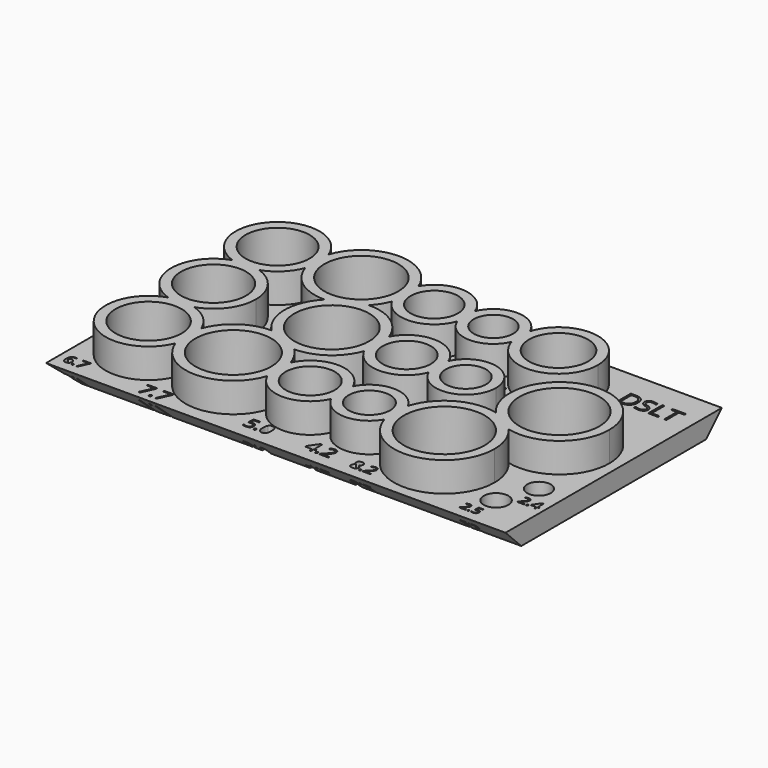
from build123d import *

# Parameters (mm, degrees)
F0_R         = 3.25
F0_R_2       = 3.3
F0_R_3       = 3.35
F0_R_4       = 3.85
F0_R_5       = 3.8
F0_R_6       = 3.75
F0_R_7       = 2.4
F0_R_8       = 2
F0_R_9       = 2.45
F0_R_10      = 2.5
F0_R_11      = 2.1
F0_R_12      = 2.05
F0_R_13      = 4.1
F0_R_14      = 4.05
F0_R_15      = 3
F1_DEPTH     = 5
F0_W         = 46.6128331609
F0_H         = 27.4442788213
F0_R_16      = 1.25
F0_R_17      = 1.2
F2_DEPTH     = 2
F3_TEXT_SIZE = 2.4939923362
F4_DEPTH     = 1
F5_T1_DEPTH  = 56.8995651128
F5_T3_DEPTH  = 37.7310107732


# Not quite as in the source:
# - a fillet or chamfer that OpenCascade refuses, or shapes differently, is made with other operations: its cross-section is extruded or revolved along the edge and cut away or added
# - Text() gives the source's letters only with a copy of the font that has no kerning and outlines rounded to 1/6400 em; it was checked with that copy


with BuildPart() as f1:
    # F0 (on Top) → F1 (new body)
    with BuildSketch(Plane.XY):
        with BuildLine():
            ThreePointArc((3.9852941176, 6.6460001836), (3.75, 8.122459054), (3.9852941176, 9.5989179243))
            ThreePointArc((3.9852941176, 9.5989179243), (-3.0577682778, 11.0741624875), (-1.3349053155, 4.0875454491))
            ThreePointArc((-1.3349053155, 4.0875454491), (0, 4.3), (1.3349053155, 4.0875454491))
            ThreePointArc((1.3349053155, 4.0875454491), (2.9517034335, 5.0646907762), (3.9852941176, 6.6460001836))
        make_face()
        with Locations((0, 8.122459054)):
            Circle(F0_R, mode=Mode.SUBTRACT)
        with BuildLine():
            ThreePointArc((1.3349053155, 4.0875454491), (0, 4.3), (-1.3349053155, 4.0875454491))
            ThreePointArc((-1.3349053155, 4.0875454491), (0, 3.872459054), (1.3349053155, 4.0875454491))
        make_face()
        with BuildLine():
            ThreePointArc((1.3349053155, 4.0875454491), (0, 3.872459054), (-1.3349053155, 4.0875454491))
            ThreePointArc((-1.3349053155, 4.0875454491), (-4.299991628, -0.0084852232), (-1.3187629808, -4.0927819635))
            ThreePointArc((-1.3187629808, -4.0927819635), (0, -3.8880641252), (1.3187629808, -4.0927819635))
            ThreePointArc((1.3187629808, -4.0927819635), (3.4756784099, -2.5317305526), (4.3, 0))
            ThreePointArc((4.3, 0), (3.4806675262, 2.5248670404), (1.3349053155, 4.0875454491))
        make_face()
        Circle(F0_R_2, mode=Mode.SUBTRACT)
        with BuildLine():
            ThreePointArc((1.3187629808, -4.0927819635), (0, -3.8880641252), (-1.3187629808, -4.0927819635))
            ThreePointArc((-1.3187629808, -4.0927819635), (0, -4.3), (1.3187629808, -4.0927819635))
        make_face()
        with BuildLine():
            ThreePointArc((1.3187629808, -4.0927819635), (0, -4.3), (-1.3187629808, -4.0927819635))
            ThreePointArc((-1.3187629808, -4.0927819635), (-3.191120568, -11.1942862955), (4.0325581395, -9.8693136007))
            ThreePointArc((4.0325581395, -9.8693136007), (3.75, -8.2380641252), (4.0325581395, -6.6068146497))
            ThreePointArc((4.0325581395, -6.6068146497), (2.9562221703, -5.0469435571), (1.3187629808, -4.0927819635))
        make_face()
        with Locations((0, -8.2380641252)):
            Circle(F0_R_3, mode=Mode.SUBTRACT)
        with BuildLine():
            ThreePointArc((12.0208047361, -4.7999549126), (10.1687837758, -4.4369637299), (8.5998497874, -3.3880641275))
            ThreePointArc((8.5998497874, -3.3880641275), (5.8061114791, -4.2736364322), (4.0325581395, -6.6068146497))
            ThreePointArc((4.0325581395, -6.6068146497), (4.2699021012, -7.4071393112), (4.35, -8.2380641252))
            ThreePointArc((4.35, -8.2380641252), (4.2699021012, -9.0689889392), (4.0325581395, -9.8693136007))
            ThreePointArc((4.0325581395, -9.8693136007), (8.6863057304, -13.0872961593), (13.2225961538, -9.7057510122))
            ThreePointArc((13.2225961538, -9.7057510122), (12.9, -8.2380641252), (13.2225961538, -6.7703772381))
            ThreePointArc((13.2225961538, -6.7703772381), (12.7406177684, -5.7126365385), (12.0208047361, -4.7999549126))
        make_face()
        with Locations((8.6, -8.2380641252)):
            Circle(F0_R_4, mode=Mode.SUBTRACT)
        with BuildLine():
            ThreePointArc((16.5327302632, 1.5793531465), (14.7366295871, 3.9434576837), (11.8935105964, 4.7988186053))
            ThreePointArc((11.8935105964, 4.7988186053), (10.3797093305, 3.7602127482), (8.5851245704, 3.3732218723))
            ThreePointArc((8.5851245704, 3.3732218723), (7.2000113835, -0.010453762), (8.5998497874, -3.3880641275))
            ThreePointArc((8.5998497874, -3.3880641275), (10.4502913932, -3.7548820231), (12.0208047361, -4.7999549126))
            ThreePointArc((12.0208047361, -4.7999549126), (14.7886805448, -3.9068223429), (16.5327302632, -1.5793531465))
            ThreePointArc((16.5327302632, -1.5793531465), (16.15, 0), (16.5327302632, 1.5793531465))
        make_face()
        with Locations((12, 0)):
            Circle(F0_R_5, mode=Mode.SUBTRACT)
        with BuildLine():
            ThreePointArc((12.9434121622, 6.4435938548), (12.5, 8.122459054), (12.9434121622, 9.8013242532))
            ThreePointArc((12.9434121622, 9.8013242532), (8.3927023806, 12.8712470279), (3.9852941176, 9.5989179243))
            ThreePointArc((3.9852941176, 9.5989179243), (4.1833001327, 8.872459054), (4.25, 8.122459054))
            ThreePointArc((4.25, 8.122459054), (4.1833001327, 7.372459054), (3.9852941176, 6.6460001836))
            ThreePointArc((3.9852941176, 6.6460001836), (5.7462630629, 4.2521318222), (8.5851245704, 3.3732218723))
            ThreePointArc((8.5851245704, 3.3732218723), (10.1005042555, 4.408164688), (11.8935105964, 4.7988186053))
            ThreePointArc((11.8935105964, 4.7988186053), (12.5038307889, 5.5667127807), (12.9434121622, 6.4435938548))
        make_face()
        with Locations((8.5, 8.122459054)):
            Circle(F0_R_6, mode=Mode.SUBTRACT)
        with BuildLine():
            ThreePointArc((13.25, 8.122459054), (13.1727244606, 8.9757738346), (12.9434121622, 9.8013242532))
            ThreePointArc((12.9434121622, 9.8013242532), (12.5, 8.122459054), (12.9434121622, 6.4435938548))
            ThreePointArc((12.9434121622, 6.4435938548), (13.1727244606, 7.2691442733), (13.25, 8.122459054))
        make_face()
        with BuildLine():
            ThreePointArc((19.1133333333, 7.011383499), (18.9, 8.122459054), (19.1133333333, 9.233534609))
            ThreePointArc((19.1133333333, 9.233534609), (16.2115699478, 11.5081530992), (12.9434121622, 9.8013242532))
            ThreePointArc((12.9434121622, 9.8013242532), (13.1727244606, 8.9757738346), (13.25, 8.122459054))
            ThreePointArc((13.25, 8.122459054), (13.1727244606, 7.2691442733), (12.9434121622, 6.4435938548))
            ThreePointArc((12.9434121622, 6.4435938548), (16.2115699478, 4.7367650088), (19.1133333333, 7.011383499))
        make_face()
        with Locations((15.9, 8.122459054)):
            Circle(F0_R_7, mode=Mode.SUBTRACT)
        with BuildLine():
            ThreePointArc((19.3, 8.122459054), (19.2530085993, 8.6857825253), (19.1133333333, 9.233534609))
            ThreePointArc((19.1133333333, 9.233534609), (18.9, 8.122459054), (19.1133333333, 7.011383499))
            ThreePointArc((19.1133333333, 7.011383499), (19.2530085993, 7.5591355827), (19.3, 8.122459054))
        make_face()
        with BuildLine():
            ThreePointArc((24.6696969697, 6.9697324186), (24.5, 8.122459054), (24.6696969697, 9.2751856894))
            ThreePointArc((24.6696969697, 9.2751856894), (21.8775123194, 11.1223747702), (19.1133333333, 9.233534609))
            ThreePointArc((19.1133333333, 9.233534609), (19.2530085993, 8.6857825253), (19.3, 8.122459054))
            ThreePointArc((19.3, 8.122459054), (19.2530085993, 7.5591355827), (19.1133333333, 7.011383499))
            ThreePointArc((19.1133333333, 7.011383499), (21.8775123194, 5.1225433378), (24.6696969697, 6.9697324186))
        make_face()
        with Locations((21.9, 8.122459054)):
            Circle(F0_R_8, mode=Mode.SUBTRACT)
        with BuildLine():
            ThreePointArc((22.8166666667, 1.2472191289), (19.7820936904, 3.445191125), (16.5327302632, 1.5793531465))
            ThreePointArc((16.5327302632, 1.5793531465), (16.7327109178, 0.8009040944), (16.8, 0))
            ThreePointArc((16.8, 0), (16.7327109178, -0.8009040944), (16.5327302632, -1.5793531465))
            ThreePointArc((16.5327302632, -1.5793531465), (19.7820936904, -3.445191125), (22.8166666667, -1.2472191289))
            ThreePointArc((22.8166666667, -1.2472191289), (22.55, 0), (22.8166666667, 1.2472191289))
        make_face()
        with Locations((19.6, 0)):
            Circle(F0_R_9, mode=Mode.SUBTRACT)
        with BuildLine():
            ThreePointArc((16.8, 0), (16.7327109178, 0.8009040944), (16.5327302632, 1.5793531465))
            ThreePointArc((16.5327302632, 1.5793531465), (16.15, 0), (16.5327302632, -1.5793531465))
            ThreePointArc((16.5327302632, -1.5793531465), (16.7327109178, -0.8009040944), (16.8, 0))
        make_face()
        with BuildLine():
            ThreePointArc((13.2225961538, -6.7703772381), (12.9, -8.2380641252), (13.2225961538, -9.7057510122))
            ThreePointArc((13.2225961538, -9.7057510122), (13.3928118754, -8.9806638336), (13.45, -8.2380641252))
            ThreePointArc((13.45, -8.2380641252), (13.3928118754, -7.4954644168), (13.2225961538, -6.7703772381))
        make_face()
        with BuildLine():
            ThreePointArc((13.45, -8.2380641252), (13.3928118754, -8.9806638336), (13.2225961538, -9.7057510122))
            ThreePointArc((13.2225961538, -9.7057510122), (16.4525004244, -11.7376703467), (19.62, -9.6097783811))
            ThreePointArc((19.62, -9.6097783811), (19.3, -8.2380641252), (19.62, -6.8663498692))
            ThreePointArc((19.62, -6.8663498692), (16.4525004244, -4.7384579037), (13.2225961538, -6.7703772381))
            ThreePointArc((13.2225961538, -6.7703772381), (13.3928118754, -7.4954644168), (13.45, -8.2380641252))
        make_face()
        with Locations((16.4, -8.2380641252)):
            Circle(F0_R_10, mode=Mode.SUBTRACT)
        with BuildLine():
            ThreePointArc((19.62, -6.8663498692), (19.3, -8.2380641252), (19.62, -9.6097783811))
            ThreePointArc((19.62, -9.6097783811), (19.8292856399, -8.9380641252), (19.9, -8.2380641252))
            ThreePointArc((19.9, -8.2380641252), (19.8292856399, -7.5380641252), (19.62, -6.8663498692))
        make_face()
        with BuildLine():
            ThreePointArc((19.9, -8.2380641252), (19.8292856399, -8.9380641252), (19.62, -9.6097783811))
            ThreePointArc((19.62, -9.6097783811), (22.336051002, -11.3374044624), (25.1210526316, -9.7232821483))
            ThreePointArc((25.1210526316, -9.7232821483), (24.9, -8.2380641252), (25.1210526316, -6.7528461021))
            ThreePointArc((25.1210526316, -6.7528461021), (22.336051002, -5.138723788), (19.62, -6.8663498692))
            ThreePointArc((19.62, -6.8663498692), (19.8292856399, -7.5380641252), (19.9, -8.2380641252))
        make_face()
        with Locations((22.4, -8.2380641252)):
            Circle(F0_R_11, mode=Mode.SUBTRACT)
        with BuildLine():
            ThreePointArc((23.05, 0), (22.9911649916, 0.634428877), (22.8166666667, 1.2472191289))
            ThreePointArc((22.8166666667, 1.2472191289), (22.55, 0), (22.8166666667, -1.2472191289))
            ThreePointArc((22.8166666667, -1.2472191289), (22.9911649916, -0.634428877), (23.05, 0))
        make_face()
        with BuildLine():
            ThreePointArc((28.65, 0), (26.2377042157, 2.9825883614), (22.8166666667, 1.2472191289))
            ThreePointArc((22.8166666667, 1.2472191289), (22.9911649916, 0.634428877), (23.05, 0))
            ThreePointArc((23.05, 0), (22.9911649916, -0.634428877), (22.8166666667, -1.2472191289))
            ThreePointArc((22.8166666667, -1.2472191289), (26.2377042157, -2.9825883614), (28.65, 0))
        make_face()
        with Locations((25.6, 0)):
            Circle(F0_R_12, mode=Mode.SUBTRACT)
        with BuildLine():
            ThreePointArc((25.5, -8.2380641252), (25.4037695616, -9.0044637736), (25.1210526316, -9.7232821483))
            ThreePointArc((25.1210526316, -9.7232821483), (30.7507890586, -13.2824982649), (35.1, -8.2380641252))
            ThreePointArc((35.1, -8.2380641252), (34.7771588225, -6.4523559787), (33.8495083983, -4.892726311))
            ThreePointArc((33.8495083983, -4.892726311), (32.4418164946, -4.2937816027), (31.2780626343, -3.3008021407))
            ThreePointArc((31.2780626343, -3.3008021407), (27.5058579441, -3.7895525308), (25.1210526316, -6.7528461021))
            ThreePointArc((25.1210526316, -6.7528461021), (25.4037695616, -7.4716644768), (25.5, -8.2380641252))
        make_face()
        with Locations((30, -8.2380641252)):
            Circle(F0_R_13, mode=Mode.SUBTRACT)
        with BuildLine():
            ThreePointArc((25.1210526316, -6.7528461021), (24.9, -8.2380641252), (25.1210526316, -9.7232821483))
            ThreePointArc((25.1210526316, -9.7232821483), (25.4037695616, -9.0044637736), (25.5, -8.2380641252))
            ThreePointArc((25.5, -8.2380641252), (25.4037695616, -7.4716644768), (25.1210526316, -6.7528461021))
        make_face()
        with BuildLine():
            ThreePointArc((33.8495083983, -4.892726311), (32.6845021539, -3.9017698333), (31.2780626343, -3.3008021407))
            ThreePointArc((31.2780626343, -3.3008021407), (32.4418164946, -4.2937816027), (33.8495083983, -4.892726311))
        make_face()
        with BuildLine():
            ThreePointArc((40.15, 0), (33.339074632, 4.7330372752), (31.2780626343, -3.3008021407))
            ThreePointArc((31.2780626343, -3.3008021407), (32.6845021539, -3.9017698333), (33.8495083983, -4.892726311))
            ThreePointArc((33.8495083983, -4.892726311), (38.1973793287, -3.9885763493), (40.15, 0))
        make_face()
        with Locations((35.1, 0)):
            Circle(F0_R_14, mode=Mode.SUBTRACT)
        with BuildLine():
            ThreePointArc((24.9, 8.122459054), (24.8418608829, 8.7102128676), (24.6696969697, 9.2751856894))
            ThreePointArc((24.6696969697, 9.2751856894), (24.5, 8.122459054), (24.6696969697, 6.9697324186))
            ThreePointArc((24.6696969697, 6.9697324186), (24.8418608829, 7.5347052403), (24.9, 8.122459054))
        make_face()
        with BuildLine():
            ThreePointArc((24.6696969697, 6.9697324186), (29.082575265, 4.1651106917), (32.5, 8.122459054))
            ThreePointArc((32.5, 8.122459054), (29.082575265, 12.0798074163), (24.6696969697, 9.2751856894))
            ThreePointArc((24.6696969697, 9.2751856894), (24.8418608829, 8.7102128676), (24.9, 8.122459054))
            ThreePointArc((24.9, 8.122459054), (24.8418608829, 7.5347052403), (24.6696969697, 6.9697324186))
        make_face()
        with Locations((28.5, 8.122459054)):
            Circle(F0_R_15, mode=Mode.SUBTRACT)
        with BuildLine():
            ThreePointArc((4.25, 8.122459054), (4.1833001327, 8.872459054), (3.9852941176, 9.5989179243))
            ThreePointArc((3.9852941176, 9.5989179243), (3.75, 8.122459054), (3.9852941176, 6.6460001836))
            ThreePointArc((3.9852941176, 6.6460001836), (4.1833001327, 7.372459054), (4.25, 8.122459054))
        make_face()
        with BuildLine():
            ThreePointArc((4.0325581395, -6.6068146497), (3.75, -8.2380641252), (4.0325581395, -9.8693136007))
            ThreePointArc((4.0325581395, -9.8693136007), (4.2699021012, -9.0689889392), (4.35, -8.2380641252))
            ThreePointArc((4.35, -8.2380641252), (4.2699021012, -7.4071393112), (4.0325581395, -6.6068146497))
        make_face()
        with BuildLine():
            ThreePointArc((12.0208047361, -4.7999549126), (10.4502913932, -3.7548820231), (8.5998497874, -3.3880641275))
            ThreePointArc((8.5998497874, -3.3880641275), (10.1687837758, -4.4369637299), (12.0208047361, -4.7999549126))
        make_face()
        with BuildLine():
            ThreePointArc((8.5851245704, 3.3732218723), (10.3797093305, 3.7602127482), (11.8935105964, 4.7988186053))
            ThreePointArc((11.8935105964, 4.7988186053), (10.1005042555, 4.408164688), (8.5851245704, 3.3732218723))
        make_face()
    extrude(amount=F1_DEPTH)

    # F0 (on Top) → F2 (join)
    with BuildSketch(Plane.XY):
        with Locations((17.849897733, -0.6956402212)):
            Rectangle(F0_W, F0_H)
        with BuildLine():
            add(Edge.make_bspline(
                [(-4.5829944917, -13.2263076646), (-4.683570923, -13.0972890416), (-4.683570923, -12.8673308955)],
                knots=[0, 0, 0, 1, 1, 1], degree=2))
            add(Edge.make_bspline(
                [(-4.683570923, -12.8673308955), (-4.683570923, -12.5412744504), (-4.5568518814, -12.3798196257)],
                knots=[0, 0, 0, 1, 1, 1], degree=2))
            add(Edge.make_bspline(
                [(-4.5568518814, -12.3798196257), (-4.4301328398, -12.218364801), (-4.1820201032, -12.218364801)],
                knots=[0, 0, 0, 1, 1, 1], degree=2))
            add(Edge.make_bspline(
                [(-4.1820201032, -12.218364801), (-4.0965724974, -12.218364801), (-4.0474340725, -12.2326464122)],
                knots=[0, 0, 0, 1, 1, 1], degree=2))
            Line((-4.0474340725, -12.2326464122), (-4.0474340725, -12.3408477715))
            add(Edge.make_bspline(
                [(-4.0474340725, -12.3408477715), (-4.1057708232, -12.3219669974), (-4.180567736, -12.3219669974)],
                knots=[0, 0, 0, 1, 1, 1], degree=2))
            add(Edge.make_bspline(
                [(-4.180567736, -12.3219669974), (-4.3584827227, -12.3219669974), (-4.4522814402, -12.4327099993)],
                knots=[0, 0, 0, 1, 1, 1], degree=2))
            add(Edge.make_bspline(
                [(-4.4522814402, -12.4327099993), (-4.5460801577, -12.5434530012), (-4.5550364224, -12.781157106)],
                knots=[0, 0, 0, 1, 1, 1], degree=2))
            Line((-4.5550364224, -12.781157106), (-4.5460801577, -12.781157106))
            add(Edge.make_bspline(
                [(-4.5460801577, -12.781157106), (-4.4628111027, -12.6509281769), (-4.2827175651, -12.6509281769)],
                knots=[0, 0, 0, 1, 1, 1], degree=2))
            add(Edge.make_bspline(
                [(-4.2827175651, -12.6509281769), (-4.133607862, -12.6509281769), (-4.0477971643, -12.7409749457)],
                knots=[0, 0, 0, 1, 1, 1], degree=2))
            add(Edge.make_bspline(
                [(-4.0477971643, -12.7409749457), (-3.9619864666, -12.8310217145), (-3.9619864666, -12.985214703)],
                knots=[0, 0, 0, 1, 1, 1], degree=2))
            add(Edge.make_bspline(
                [(-3.9619864666, -12.985214703), (-3.9619864666, -13.1578043432), (-4.0561482759, -13.2565653154)],
                knots=[0, 0, 0, 1, 1, 1], degree=2))
            add(Edge.make_bspline(
                [(-4.0561482759, -13.2565653154), (-4.1503100852, -13.3553262876), (-4.3107966651, -13.3553262876)],
                knots=[0, 0, 0, 1, 1, 1], degree=2))
            add(Edge.make_bspline(
                [(-4.3107966651, -13.3553262876), (-4.4824180604, -13.3553262876), (-4.5829944917, -13.2263076646)],
                knots=[0, 0, 0, 1, 1, 1], degree=2))
        make_face(mode=Mode.SUBTRACT)
        with BuildLine():
            add(Edge.make_bspline(
                [(-3.7461889011, -13.3382609726), (-3.7714842971, -13.3144179437), (-3.7714842971, -13.2599541723)],
                knots=[0, 0, 0, 1, 1, 1], degree=2))
            add(Edge.make_bspline(
                [(-3.7714842971, -13.2599541723), (-3.7714842971, -13.2091213189), (-3.7483674519, -13.1830997393)],
                knots=[0, 0, 0, 1, 1, 1], degree=2))
            add(Edge.make_bspline(
                [(-3.7483674519, -13.1830997393), (-3.7252506067, -13.1570781596), (-3.682163712, -13.1570781596)],
                knots=[0, 0, 0, 1, 1, 1], degree=2))
            add(Edge.make_bspline(
                [(-3.682163712, -13.1570781596), (-3.6383506336, -13.1570781596), (-3.6137814211, -13.1830997393)],
                knots=[0, 0, 0, 1, 1, 1], degree=2))
            add(Edge.make_bspline(
                [(-3.6137814211, -13.1830997393), (-3.5892122087, -13.2091213189), (-3.5892122087, -13.2599541723)],
                knots=[0, 0, 0, 1, 1, 1], degree=2))
            add(Edge.make_bspline(
                [(-3.5892122087, -13.2599541723), (-3.5892122087, -13.3090925972), (-3.6141445129, -13.3355982993)],
                knots=[0, 0, 0, 1, 1, 1], degree=2))
            add(Edge.make_bspline(
                [(-3.6141445129, -13.3355982993), (-3.6390768172, -13.3621040014), (-3.682163712, -13.3621040014)],
                knots=[0, 0, 0, 1, 1, 1], degree=2))
            add(Edge.make_bspline(
                [(-3.682163712, -13.3621040014), (-3.720893505, -13.3621040014), (-3.7461889011, -13.3382609726)],
                knots=[0, 0, 0, 1, 1, 1], degree=2))
        make_face(mode=Mode.SUBTRACT)
        Polygon((-3.119371407, -13.3400764316), (-3.2585566007, -13.3400764316), (-2.8003347369, -12.3498040361), (-3.4030671409, -12.3498040361), (-3.4030671409, -12.2340987794), (-2.6672010734, -12.2340987794), (-2.6672010734, -12.3347962413), align=None, mode=Mode.SUBTRACT)
        with BuildLine():
            add(Edge.make_bspline(
                [(4.398838388, -13.7299771017), (4.3660354925, -13.699057626), (4.3660354925, -13.628429382)],
                knots=[0, 0, 0, 1, 1, 1], degree=2))
            add(Edge.make_bspline(
                [(4.3660354925, -13.628429382), (4.3660354925, -13.5625096876), (4.3960132583, -13.5287650821)],
                knots=[0, 0, 0, 1, 1, 1], degree=2))
            add(Edge.make_bspline(
                [(4.3960132583, -13.5287650821), (4.4259910241, -13.4950204767), (4.4818658126, -13.4950204767)],
                knots=[0, 0, 0, 1, 1, 1], degree=2))
            add(Edge.make_bspline(
                [(4.4818658126, -13.4950204767), (4.5386823111, -13.4950204767), (4.5705434968, -13.5287650821)],
                knots=[0, 0, 0, 1, 1, 1], degree=2))
            add(Edge.make_bspline(
                [(4.5705434968, -13.5287650821), (4.6024046824, -13.5625096876), (4.6024046824, -13.628429382)],
                knots=[0, 0, 0, 1, 1, 1], degree=2))
            add(Edge.make_bspline(
                [(4.6024046824, -13.628429382), (4.6024046824, -13.6921517533), (4.5700726418, -13.7265241653)],
                knots=[0, 0, 0, 1, 1, 1], degree=2))
            add(Edge.make_bspline(
                [(4.5700726418, -13.7265241653), (4.5377406012, -13.7608965774), (4.4818658126, -13.7608965774)],
                knots=[0, 0, 0, 1, 1, 1], degree=2))
            add(Edge.make_bspline(
                [(4.4818658126, -13.7608965774), (4.4316412836, -13.7608965774), (4.398838388, -13.7299771017)],
                knots=[0, 0, 0, 1, 1, 1], degree=2))
        make_face(mode=Mode.SUBTRACT)
        Polygon((3.5285414703, -13.7323313765), (3.348047069, -13.7323313765), (3.9422660285, -12.448152949), (3.1606467949, -12.448152949), (3.1606467949, -12.2981071684), (4.1149128472, -12.2981071684), (4.1149128472, -12.428690944), align=None, mode=Mode.SUBTRACT)
        Polygon((5.2116910006, -13.7323313765), (5.0311965993, -13.7323313765), (5.6254155588, -12.448152949), (4.8437963252, -12.448152949), (4.8437963252, -12.2981071684), (5.7980623774, -12.2981071684), (5.7980623774, -12.428690944), align=None, mode=Mode.SUBTRACT)
        with BuildLine():
            add(Edge.make_bspline(
                [(14.4671539264, -13.0317730066), (14.4364999457, -13.0028790631), (14.4364999457, -12.9368776692)],
                knots=[0, 0, 0, 1, 1, 1], degree=2))
            add(Edge.make_bspline(
                [(14.4364999457, -12.9368776692), (14.4364999457, -12.8752763683), (14.4645138706, -12.843742369)],
                knots=[0, 0, 0, 1, 1, 1], degree=2))
            add(Edge.make_bspline(
                [(14.4645138706, -12.843742369), (14.4925277956, -12.8122083697), (14.5447422316, -12.8122083697)],
                knots=[0, 0, 0, 1, 1, 1], degree=2))
            add(Edge.make_bspline(
                [(14.5447422316, -12.8122083697), (14.5978366862, -12.8122083697), (14.6276106484, -12.843742369)],
                knots=[0, 0, 0, 1, 1, 1], degree=2))
            add(Edge.make_bspline(
                [(14.6276106484, -12.843742369), (14.6573846105, -12.8752763683), (14.6573846105, -12.9368776692)],
                knots=[0, 0, 0, 1, 1, 1], degree=2))
            add(Edge.make_bspline(
                [(14.6573846105, -12.9368776692), (14.6573846105, -12.9964255935), (14.6271706391, -13.0285462718)],
                knots=[0, 0, 0, 1, 1, 1], degree=2))
            add(Edge.make_bspline(
                [(14.6271706391, -13.0285462718), (14.5969566676, -13.0606669502), (14.5447422316, -13.0606669502)],
                knots=[0, 0, 0, 1, 1, 1], degree=2))
            add(Edge.make_bspline(
                [(14.5447422316, -13.0606669502), (14.4978079071, -13.0606669502), (14.4671539264, -13.0317730066)],
                knots=[0, 0, 0, 1, 1, 1], degree=2))
        make_face(mode=Mode.SUBTRACT)
        with BuildLine():
            add(Edge.make_bspline(
                [(13.5245073523, -12.2363828757), (13.6298162429, -12.2152624297), (13.7345384545, -12.2152624297)],
                knots=[0, 0, 0, 1, 1, 1], degree=2))
            add(Edge.make_bspline(
                [(13.7345384545, -12.2152624297), (13.9463295939, -12.2152624297), (14.0677721586, -12.3202779808)],
                knots=[0, 0, 0, 1, 1, 1], degree=2))
            add(Edge.make_bspline(
                [(14.0677721586, -12.3202779808), (14.1892147233, -12.4252935319), (14.1892147233, -12.6077507185)],
                knots=[0, 0, 0, 1, 1, 1], degree=2))
            add(Edge.make_bspline(
                [(14.1892147233, -12.6077507185), (14.1892147233, -12.8157284441), (14.0567719263, -12.9340909437)],
                knots=[0, 0, 0, 1, 1, 1], degree=2))
            add(Edge.make_bspline(
                [(14.0567719263, -12.9340909437), (13.9243291293, -13.0524534434), (13.6914175439, -13.0524534434)],
                knots=[0, 0, 0, 1, 1, 1], degree=2))
            add(Edge.make_bspline(
                [(13.6914175439, -13.0524534434), (13.464959428, -13.0524534434), (13.3458635796, -12.9799985799)],
                knots=[0, 0, 0, 1, 1, 1], degree=2))
            Line((13.3458635796, -12.9799985799), (13.3458635796, -12.8333288158))
            add(Edge.make_bspline(
                [(13.3458635796, -12.8333288158), (13.4098115967, -12.8743963497), (13.5051469434, -12.897863512)],
                knots=[0, 0, 0, 1, 1, 1], degree=2))
            add(Edge.make_bspline(
                [(13.5051469434, -12.897863512), (13.6004822901, -12.9213306742), (13.693177581, -12.9213306742)],
                knots=[0, 0, 0, 1, 1, 1], degree=2))
            add(Edge.make_bspline(
                [(13.693177581, -12.9213306742), (13.8545143216, -12.9213306742), (13.9438362079, -12.8452090667)],
                knots=[0, 0, 0, 1, 1, 1], degree=2))
            add(Edge.make_bspline(
                [(13.9438362079, -12.8452090667), (14.0331580943, -12.7690874591), (14.0331580943, -12.6250577507)],
                knots=[0, 0, 0, 1, 1, 1], degree=2))
            add(Edge.make_bspline(
                [(14.0331580943, -12.6250577507), (14.0331580943, -12.3446251617), (13.6896575067, -12.3446251617)],
                knots=[0, 0, 0, 1, 1, 1], degree=2))
            add(Edge.make_bspline(
                [(13.6896575067, -12.3446251617), (13.6025356668, -12.3446251617), (13.4567459213, -12.3713190587)],
                knots=[0, 0, 0, 1, 1, 1], degree=2))
            Line((13.4567459213, -12.3713190587), (13.3778375881, -12.3208646599))
            Line((13.3778375881, -12.3208646599), (13.428291987, -11.6937047484))
            Line((13.428291987, -11.6937047484), (14.0947593952, -11.6937047484))
            Line((14.0947593952, -11.6937047484), (14.0947593952, -11.8339210429))
            Line((14.0947593952, -11.8339210429), (13.5585347376, -11.8339210429))
            Line((13.5585347376, -11.8339210429), (13.5245073523, -12.2363828757))
        make_face(mode=Mode.SUBTRACT)
        with BuildLine():
            add(Edge.make_bspline(
                [(15.6635391924, -11.8496147077), (15.7767682504, -12.026645113), (15.7767682504, -12.3619321938)],
                knots=[0, 0, 0, 1, 1, 1], degree=2))
            add(Edge.make_bspline(
                [(15.7767682504, -12.3619321938), (15.7767682504, -12.7095395348), (15.6672059366, -12.8809964891)],
                knots=[0, 0, 0, 1, 1, 1], degree=2))
            add(Edge.make_bspline(
                [(15.6672059366, -12.8809964891), (15.5576436227, -13.0524534434), (15.3320655255, -13.0524534434)],
                knots=[0, 0, 0, 1, 1, 1], degree=2))
            add(Edge.make_bspline(
                [(15.3320655255, -13.0524534434), (15.1158742932, -13.0524534434), (15.0030852445, -12.8768897357)],
                knots=[0, 0, 0, 1, 1, 1], degree=2))
            add(Edge.make_bspline(
                [(15.0030852445, -12.8768897357), (14.8902961959, -12.701326028), (14.8902961959, -12.3619321938)],
                knots=[0, 0, 0, 1, 1, 1], degree=2))
            add(Edge.make_bspline(
                [(14.8902961959, -12.3619321938), (14.8902961959, -12.0119781366), (14.9994185004, -11.8422812195)],
                knots=[0, 0, 0, 1, 1, 1], degree=2))
            add(Edge.make_bspline(
                [(14.9994185004, -11.8422812195), (15.108540805, -11.6725843024), (15.3320655255, -11.6725843024)],
                knots=[0, 0, 0, 1, 1, 1], degree=2))
            add(Edge.make_bspline(
                [(15.3320655255, -11.6725843024), (15.5503101345, -11.6725843024), (15.6635391924, -11.8496147077)],
                knots=[0, 0, 0, 1, 1, 1], degree=2))
        make_face(mode=Mode.SUBTRACT)
        with BuildLine():
            add(Edge.make_bspline(
                [(-3.6198314493, -4.3217159205), (-3.6423567719, -4.3004839179), (-3.6423567719, -4.2519844194)],
                knots=[0, 0, 0, 1, 1, 1], degree=2))
            add(Edge.make_bspline(
                [(-3.6423567719, -4.2519844194), (-3.6423567719, -4.2067182209), (-3.6217714292, -4.1835462383)],
                knots=[0, 0, 0, 1, 1, 1], degree=2))
            add(Edge.make_bspline(
                [(-3.6217714292, -4.1835462383), (-3.6011860865, -4.1603742557), (-3.5628175944, -4.1603742557)],
                knots=[0, 0, 0, 1, 1, 1], degree=2))
            add(Edge.make_bspline(
                [(-3.5628175944, -4.1603742557), (-3.5238024423, -4.1603742557), (-3.5019237797, -4.1835462383)],
                knots=[0, 0, 0, 1, 1, 1], degree=2))
            add(Edge.make_bspline(
                [(-3.5019237797, -4.1835462383), (-3.4800451171, -4.2067182209), (-3.4800451171, -4.2519844194)],
                knots=[0, 0, 0, 1, 1, 1], degree=2))
            add(Edge.make_bspline(
                [(-3.4800451171, -4.2519844194), (-3.4800451171, -4.2957417447), (-3.5022471097, -4.319344834)],
                knots=[0, 0, 0, 1, 1, 1], degree=2))
            add(Edge.make_bspline(
                [(-3.5022471097, -4.319344834), (-3.5244491023, -4.3429479232), (-3.5628175944, -4.3429479232)],
                knots=[0, 0, 0, 1, 1, 1], degree=2))
            add(Edge.make_bspline(
                [(-3.5628175944, -4.3429479232), (-3.5973061267, -4.3429479232), (-3.6198314493, -4.3217159205)],
                knots=[0, 0, 0, 1, 1, 1], degree=2))
        make_face(mode=Mode.SUBTRACT)
        with BuildLine():
            add(Edge.make_bspline(
                [(-4.364999299, -4.222022507), (-4.4545617061, -4.107132584), (-4.4545617061, -3.9023569238)],
                knots=[0, 0, 0, 1, 1, 1], degree=2))
            add(Edge.make_bspline(
                [(-4.4545617061, -3.9023569238), (-4.4545617061, -3.6120065931), (-4.3417195397, -3.4682325243)],
                knots=[0, 0, 0, 1, 1, 1], degree=2))
            add(Edge.make_bspline(
                [(-4.3417195397, -3.4682325243), (-4.2288773733, -3.3244584555), (-4.0079352136, -3.3244584555)],
                knots=[0, 0, 0, 1, 1, 1], degree=2))
            add(Edge.make_bspline(
                [(-4.0079352136, -3.3244584555), (-3.9318448894, -3.3244584555), (-3.8880875641, -3.3371761018)],
                knots=[0, 0, 0, 1, 1, 1], degree=2))
            Line((-3.8880875641, -3.3371761018), (-3.8880875641, -3.4335284387))
            add(Edge.make_bspline(
                [(-3.8880875641, -3.4335284387), (-3.9400359158, -3.4167152792), (-4.0066418937, -3.4167152792)],
                knots=[0, 0, 0, 1, 1, 1], degree=2))
            add(Edge.make_bspline(
                [(-4.0066418937, -3.4167152792), (-4.1650735887, -3.4167152792), (-4.2486005027, -3.5153309261)],
                knots=[0, 0, 0, 1, 1, 1], degree=2))
            add(Edge.make_bspline(
                [(-4.2486005027, -3.5153309261), (-4.3321274167, -3.613946573), (-4.3401028898, -3.8256199396)],
                knots=[0, 0, 0, 1, 1, 1], degree=2))
            Line((-4.3401028898, -3.8256199396), (-4.3321274167, -3.8256199396))
            add(Edge.make_bspline(
                [(-4.3321274167, -3.8256199396), (-4.2579770724, -3.70965225), (-4.0976053975, -3.70965225)],
                knots=[0, 0, 0, 1, 1, 1], degree=2))
            add(Edge.make_bspline(
                [(-4.0976053975, -3.70965225), (-3.9648245483, -3.70965225), (-3.8884108941, -3.7898380874)],
                knots=[0, 0, 0, 1, 1, 1], degree=2))
            add(Edge.make_bspline(
                [(-3.8884108941, -3.7898380874), (-3.8119972399, -3.8700239249), (-3.8119972399, -4.0073313938)],
                knots=[0, 0, 0, 1, 1, 1], degree=2))
            add(Edge.make_bspline(
                [(-3.8119972399, -4.0073313938), (-3.8119972399, -4.1610209156), (-3.8958474839, -4.2489666729)],
                knots=[0, 0, 0, 1, 1, 1], degree=2))
            add(Edge.make_bspline(
                [(-3.8958474839, -4.2489666729), (-3.9796977279, -4.3369124301), (-4.1226095833, -4.3369124301)],
                knots=[0, 0, 0, 1, 1, 1], degree=2))
            add(Edge.make_bspline(
                [(-4.1226095833, -4.3369124301), (-4.2754368918, -4.3369124301), (-4.364999299, -4.222022507)],
                knots=[0, 0, 0, 1, 1, 1], degree=2))
        make_face(mode=Mode.SUBTRACT)
        with BuildLine():
            add(Edge.make_bspline(
                [(-3.2092023623, -4.222022507), (-3.2987647695, -4.107132584), (-3.2987647695, -3.9023569238)],
                knots=[0, 0, 0, 1, 1, 1], degree=2))
            add(Edge.make_bspline(
                [(-3.2987647695, -3.9023569238), (-3.2987647695, -3.6120065931), (-3.1859226031, -3.4682325243)],
                knots=[0, 0, 0, 1, 1, 1], degree=2))
            add(Edge.make_bspline(
                [(-3.1859226031, -3.4682325243), (-3.0730804366, -3.3244584555), (-2.852138277, -3.3244584555)],
                knots=[0, 0, 0, 1, 1, 1], degree=2))
            add(Edge.make_bspline(
                [(-2.852138277, -3.3244584555), (-2.7760479527, -3.3244584555), (-2.7322906274, -3.3371761018)],
                knots=[0, 0, 0, 1, 1, 1], degree=2))
            Line((-2.7322906274, -3.3371761018), (-2.7322906274, -3.4335284387))
            add(Edge.make_bspline(
                [(-2.7322906274, -3.4335284387), (-2.7842389791, -3.4167152792), (-2.850844957, -3.4167152792)],
                knots=[0, 0, 0, 1, 1, 1], degree=2))
            add(Edge.make_bspline(
                [(-2.850844957, -3.4167152792), (-3.009276652, -3.4167152792), (-3.092803566, -3.5153309261)],
                knots=[0, 0, 0, 1, 1, 1], degree=2))
            add(Edge.make_bspline(
                [(-3.092803566, -3.5153309261), (-3.17633048, -3.613946573), (-3.1843059531, -3.8256199396)],
                knots=[0, 0, 0, 1, 1, 1], degree=2))
            Line((-3.1843059531, -3.8256199396), (-3.17633048, -3.8256199396))
            add(Edge.make_bspline(
                [(-3.17633048, -3.8256199396), (-3.1021801357, -3.70965225), (-2.9418084608, -3.70965225)],
                knots=[0, 0, 0, 1, 1, 1], degree=2))
            add(Edge.make_bspline(
                [(-2.9418084608, -3.70965225), (-2.8090276117, -3.70965225), (-2.7326139574, -3.7898380874)],
                knots=[0, 0, 0, 1, 1, 1], degree=2))
            add(Edge.make_bspline(
                [(-2.7326139574, -3.7898380874), (-2.6562003032, -3.8700239249), (-2.6562003032, -4.0073313938)],
                knots=[0, 0, 0, 1, 1, 1], degree=2))
            add(Edge.make_bspline(
                [(-2.6562003032, -4.0073313938), (-2.6562003032, -4.1610209156), (-2.7400505472, -4.2489666729)],
                knots=[0, 0, 0, 1, 1, 1], degree=2))
            add(Edge.make_bspline(
                [(-2.7400505472, -4.2489666729), (-2.8239007912, -4.3369124301), (-2.9668126467, -4.3369124301)],
                knots=[0, 0, 0, 1, 1, 1], degree=2))
            add(Edge.make_bspline(
                [(-2.9668126467, -4.3369124301), (-3.1196399552, -4.3369124301), (-3.2092023623, -4.222022507)],
                knots=[0, 0, 0, 1, 1, 1], degree=2))
        make_face(mode=Mode.SUBTRACT)
        with BuildLine():
            add(Edge.make_bspline(
                [(16.7067725635, -4.2452870143), (16.6849750476, -4.2247410305), (16.6849750476, -4.17780858)],
                knots=[0, 0, 0, 1, 1, 1], degree=2))
            add(Edge.make_bspline(
                [(16.6849750476, -4.17780858), (16.6849750476, -4.1340049596), (16.7048952655, -4.1115816777)],
                knots=[0, 0, 0, 1, 1, 1], degree=2))
            add(Edge.make_bspline(
                [(16.7048952655, -4.1115816777), (16.7248154833, -4.0891583958), (16.7619442664, -4.0891583958)],
                knots=[0, 0, 0, 1, 1, 1], degree=2))
            add(Edge.make_bspline(
                [(16.7619442664, -4.0891583958), (16.7996988154, -4.0891583958), (16.8208705653, -4.1115816777)],
                knots=[0, 0, 0, 1, 1, 1], degree=2))
            add(Edge.make_bspline(
                [(16.8208705653, -4.1115816777), (16.8420423151, -4.1340049596), (16.8420423151, -4.17780858)],
                knots=[0, 0, 0, 1, 1, 1], degree=2))
            add(Edge.make_bspline(
                [(16.8420423151, -4.17780858), (16.8420423151, -4.2201520797), (16.8205576823, -4.242992539)],
                knots=[0, 0, 0, 1, 1, 1], degree=2))
            add(Edge.make_bspline(
                [(16.8205576823, -4.242992539), (16.7990730494, -4.2658329982), (16.7619442664, -4.2658329982)],
                knots=[0, 0, 0, 1, 1, 1], degree=2))
            add(Edge.make_bspline(
                [(16.7619442664, -4.2658329982), (16.7285700794, -4.2658329982), (16.7067725635, -4.2452870143)],
                knots=[0, 0, 0, 1, 1, 1], degree=2))
        make_face(mode=Mode.SUBTRACT)
        Polygon((16.5591960804, -3.9293794756), (16.5591960804, -4.0278333272), (16.417772963, -4.0278333272), (16.417772963, -4.2468514293), (16.3141043946, -4.2468514293), (16.3141043946, -4.0278333272), (15.8506203728, -4.0278333272), (15.8506203728, -3.9333426603), (16.3030491952, -3.2885950853), (16.417772963, -3.2885950853), (16.417772963, -3.9293794756), align=None, mode=Mode.SUBTRACT)
        with BuildLine():
            add(Edge.make_bspline(
                [(17.5936915828, -3.4753862381), (17.6328019582, -3.5708155541), (17.6328019582, -3.700557706)],
                knots=[0, 0, 0, 1, 1, 1], degree=2))
            add(Edge.make_bspline(
                [(17.6328019582, -3.700557706), (17.6328019582, -4.2599925155), (17.1999804707, -4.2599925155)],
                knots=[0, 0, 0, 1, 1, 1], degree=2))
            add(Edge.make_bspline(
                [(17.1999804707, -4.2599925155), (17.1242627839, -4.2599925155), (17.0800419861, -4.2468514293)],
                knots=[0, 0, 0, 1, 1, 1], degree=2))
            Line((17.0800419861, -4.2468514293), (17.0800419861, -4.1536122944))
            add(Edge.make_bspline(
                [(17.0800419861, -4.1536122944), (17.1321891533, -4.1705079766), (17.19852035, -4.1705079766)],
                knots=[0, 0, 0, 1, 1, 1], degree=2))
            add(Edge.make_bspline(
                [(17.19852035, -4.1705079766), (17.3549618515, -4.1705079766), (17.4348513116, -4.0737228343)],
                knots=[0, 0, 0, 1, 1, 1], degree=2))
            add(Edge.make_bspline(
                [(17.4348513116, -4.0737228343), (17.5147407717, -3.976937692), (17.5218327865, -3.7769011587)],
                knots=[0, 0, 0, 1, 1, 1], degree=2))
            Line((17.5218327865, -3.7769011587), (17.5141150057, -3.7769011587))
            add(Edge.make_bspline(
                [(17.5141150057, -3.7769011587), (17.4782377547, -3.8309256239), (17.4188942785, -3.8592936829)],
                knots=[0, 0, 0, 1, 1, 1], degree=2))
            add(Edge.make_bspline(
                [(17.4188942785, -3.8592936829), (17.3595508022, -3.8876617418), (17.2852932362, -3.8876617418)],
                knots=[0, 0, 0, 1, 1, 1], degree=2))
            add(Edge.make_bspline(
                [(17.2852932362, -3.8876617418), (17.1588885029, -3.8876617418), (17.0845266425, -3.8120483494)],
                knots=[0, 0, 0, 1, 1, 1], degree=2))
            add(Edge.make_bspline(
                [(17.0845266425, -3.8120483494), (17.0101647821, -3.736434957), (17.0101647821, -3.6008523224)],
                knots=[0, 0, 0, 1, 1, 1], degree=2))
            add(Edge.make_bspline(
                [(17.0101647821, -3.6008523224), (17.0101647821, -3.4523371902), (17.0932873666, -3.3662943644)],
                knots=[0, 0, 0, 1, 1, 1], degree=2))
            add(Edge.make_bspline(
                [(17.0932873666, -3.3662943644), (17.1764099511, -3.2802515386), (17.3119925857, -3.2802515386)],
                knots=[0, 0, 0, 1, 1, 1], degree=2))
            add(Edge.make_bspline(
                [(17.3119925857, -3.2802515386), (17.4091949054, -3.2802515386), (17.4818880564, -3.3301042304)],
                knots=[0, 0, 0, 1, 1, 1], degree=2))
            add(Edge.make_bspline(
                [(17.4818880564, -3.3301042304), (17.5545812075, -3.3799569222), (17.5936915828, -3.4753862381)],
                knots=[0, 0, 0, 1, 1, 1], degree=2))
        make_face(mode=Mode.SUBTRACT)
        with BuildLine():
            add(Edge.make_bspline(
                [(20.7908837508, -13.1091091359), (20.7587898597, -13.0788579562), (20.7587898597, -13.0097562768)],
                knots=[0, 0, 0, 1, 1, 1], degree=2))
            add(Edge.make_bspline(
                [(20.7587898597, -13.0097562768), (20.7587898597, -12.945261376), (20.7881196837, -12.9122461292)],
                knots=[0, 0, 0, 1, 1, 1], degree=2))
            add(Edge.make_bspline(
                [(20.7881196837, -12.9122461292), (20.8174495076, -12.8792308824), (20.8721166139, -12.8792308824)],
                knots=[0, 0, 0, 1, 1, 1], degree=2))
            add(Edge.make_bspline(
                [(20.8721166139, -12.8792308824), (20.927705076, -12.8792308824), (20.9588776114, -12.9122461292)],
                knots=[0, 0, 0, 1, 1, 1], degree=2))
            add(Edge.make_bspline(
                [(20.9588776114, -12.9122461292), (20.9900501468, -12.945261376), (20.9900501468, -13.0097562768)],
                knots=[0, 0, 0, 1, 1, 1], degree=2))
            add(Edge.make_bspline(
                [(20.9900501468, -13.0097562768), (20.9900501468, -13.0721013476), (20.9584169336, -13.1057308315)],
                knots=[0, 0, 0, 1, 1, 1], degree=2))
            add(Edge.make_bspline(
                [(20.9584169336, -13.1057308315), (20.9267837203, -13.1393603155), (20.8721166139, -13.1393603155)],
                knots=[0, 0, 0, 1, 1, 1], degree=2))
            add(Edge.make_bspline(
                [(20.8721166139, -13.1393603155), (20.8229776419, -13.1393603155), (20.7908837508, -13.1091091359)],
                knots=[0, 0, 0, 1, 1, 1], degree=2))
        make_face(mode=Mode.SUBTRACT)
        Polygon((20.5735973589, -12.6439780539), (20.5735973589, -12.7889380213), (20.365370965, -12.7889380213), (20.365370965, -13.1114125252), (20.2127330332, -13.1114125252), (20.2127330332, -12.7889380213), (19.5303155593, -12.7889380213), (19.5303155593, -12.6498133068), (20.1964557487, -11.7005097911), (20.365370965, -11.7005097911), (20.365370965, -12.6439780539), align=None, mode=Mode.SUBTRACT)
        with BuildLine():
            Line((22.1543366651, -12.9636884905), (22.1543366651, -13.1114125252))
            Line((22.1543366651, -13.1114125252), (21.232059584, -13.1114125252))
            Line((21.232059584, -13.1114125252), (21.232059584, -12.9741305221))
            Line((21.232059584, -12.9741305221), (21.6015232298, -12.6028241648))
            add(Edge.make_bspline(
                [(21.6015232298, -12.6028241648), (21.7704384462, -12.4317591184), (21.8241841968, -12.3588184569)],
                knots=[0, 0, 0, 1, 1, 1], degree=2))
            add(Edge.make_bspline(
                [(21.8241841968, -12.3588184569), (21.8779299474, -12.2858777953), (21.9048028228, -12.2167761159)],
                knots=[0, 0, 0, 1, 1, 1], degree=2))
            add(Edge.make_bspline(
                [(21.9048028228, -12.2167761159), (21.9316756981, -12.1476744365), (21.9316756981, -12.0681307255)],
                knots=[0, 0, 0, 1, 1, 1], degree=2))
            add(Edge.make_bspline(
                [(21.9316756981, -12.0681307255), (21.9316756981, -11.955725327), (21.8634953744, -11.8900019519)],
                knots=[0, 0, 0, 1, 1, 1], degree=2))
            add(Edge.make_bspline(
                [(21.8634953744, -11.8900019519), (21.7953150507, -11.8242785769), (21.6743103321, -11.8242785769)],
                knots=[0, 0, 0, 1, 1, 1], degree=2))
            add(Edge.make_bspline(
                [(21.6743103321, -11.8242785769), (21.5870886568, -11.8242785769), (21.5087734202, -11.8531477229)],
                knots=[0, 0, 0, 1, 1, 1], degree=2))
            add(Edge.make_bspline(
                [(21.5087734202, -11.8531477229), (21.4304581835, -11.882016869), (21.3346371881, -11.957875157)],
                knots=[0, 0, 0, 1, 1, 1], degree=2))
            Line((21.3346371881, -11.957875157), (21.2501795799, -11.8494623))
            add(Edge.make_bspline(
                [(21.2501795799, -11.8494623), (21.4439714008, -11.6882250481), (21.6724676207, -11.6882250481)],
                knots=[0, 0, 0, 1, 1, 1], degree=2))
            add(Edge.make_bspline(
                [(21.6724676207, -11.6882250481), (21.8702519831, -11.6882250481), (21.9825038223, -11.7894206186)],
                knots=[0, 0, 0, 1, 1, 1], degree=2))
            add(Edge.make_bspline(
                [(21.9825038223, -11.7894206186), (22.0947556615, -11.8906161891), (22.0947556615, -12.0613741169)],
                knots=[0, 0, 0, 1, 1, 1], degree=2))
            add(Edge.make_bspline(
                [(22.0947556615, -12.0613741169), (22.0947556615, -12.194970697), (22.0198187292, -12.3254960915)],
                knots=[0, 0, 0, 1, 1, 1], degree=2))
            add(Edge.make_bspline(
                [(22.0198187292, -12.3254960915), (21.9448817968, -12.4560214859), (21.7397265886, -12.6556485597)],
                knots=[0, 0, 0, 1, 1, 1], degree=2))
            Line((21.7397265886, -12.6556485597), (21.4326080135, -12.9560105262))
            Line((21.4326080135, -12.9560105262), (21.4326080135, -12.9636884905))
            Line((21.4326080135, -12.9636884905), (22.1543366651, -12.9636884905))
        make_face(mode=Mode.SUBTRACT)
        with BuildLine():
            add(Edge.make_bspline(
                [(25.3550255371, -13.271393174), (25.3276137185, -13.2455552397), (25.3276137185, -13.1865345776)],
                knots=[0, 0, 0, 1, 1, 1], degree=2))
            add(Edge.make_bspline(
                [(25.3276137185, -13.1865345776), (25.3276137185, -13.1314486264), (25.3526647106, -13.1032498656)],
                knots=[0, 0, 0, 1, 1, 1], degree=2))
            add(Edge.make_bspline(
                [(25.3526647106, -13.1032498656), (25.3777157027, -13.0750511048), (25.4244076043, -13.0750511048)],
                knots=[0, 0, 0, 1, 1, 1], degree=2))
            add(Edge.make_bspline(
                [(25.4244076043, -13.0750511048), (25.471886448, -13.0750511048), (25.4985113244, -13.1032498656)],
                knots=[0, 0, 0, 1, 1, 1], degree=2))
            add(Edge.make_bspline(
                [(25.4985113244, -13.1032498656), (25.5251362009, -13.1314486264), (25.5251362009, -13.1865345776)],
                knots=[0, 0, 0, 1, 1, 1], degree=2))
            add(Edge.make_bspline(
                [(25.5251362009, -13.1865345776), (25.5251362009, -13.2397843305), (25.4981178533, -13.2685077194)],
                knots=[0, 0, 0, 1, 1, 1], degree=2))
            add(Edge.make_bspline(
                [(25.4981178533, -13.2685077194), (25.4710995058, -13.2972311083), (25.4244076043, -13.2972311083)],
                knots=[0, 0, 0, 1, 1, 1], degree=2))
            add(Edge.make_bspline(
                [(25.4244076043, -13.2972311083), (25.3824373557, -13.2972311083), (25.3550255371, -13.271393174)],
                knots=[0, 0, 0, 1, 1, 1], degree=2))
        make_face(mode=Mode.SUBTRACT)
        with BuildLine():
            add(Edge.make_bspline(
                [(24.4640758539, -12.1351798506), (24.5603451116, -12.0577972048), (24.7219305686, -12.0577972048)],
                knots=[0, 0, 0, 1, 1, 1], degree=2))
            add(Edge.make_bspline(
                [(24.7219305686, -12.0577972048), (24.8858768521, -12.0577972048), (24.9817526387, -12.1339994374)],
                knots=[0, 0, 0, 1, 1, 1], degree=2))
            add(Edge.make_bspline(
                [(24.9817526387, -12.1339994374), (25.0776284253, -12.21020167), (25.0776284253, -12.3445064654)],
                knots=[0, 0, 0, 1, 1, 1], degree=2))
            add(Edge.make_bspline(
                [(25.0776284253, -12.3445064654), (25.0776284253, -12.4331686156), (25.0228047881, -12.5060919225)],
                knots=[0, 0, 0, 1, 1, 1], degree=2))
            add(Edge.make_bspline(
                [(25.0228047881, -12.5060919225), (24.9679811509, -12.5790152294), (24.8473166862, -12.6388228336)],
                knots=[0, 0, 0, 1, 1, 1], degree=2))
            add(Edge.make_bspline(
                [(24.8473166862, -12.6388228336), (24.9931633001, -12.7085983719), (25.0546759457, -12.7851940756)],
                knots=[0, 0, 0, 1, 1, 1], degree=2))
            add(Edge.make_bspline(
                [(25.0546759457, -12.7851940756), (25.1161885912, -12.8617897792), (25.1161885912, -12.9627806899)],
                knots=[0, 0, 0, 1, 1, 1], degree=2))
            add(Edge.make_bspline(
                [(25.1161885912, -12.9627806899), (25.1161885912, -13.1117750723), (25.0120499119, -13.2008306935)],
                knots=[0, 0, 0, 1, 1, 1], degree=2))
            add(Edge.make_bspline(
                [(25.0120499119, -13.2008306935), (24.9079112326, -13.2898863148), (24.7269145356, -13.2898863148)],
                knots=[0, 0, 0, 1, 1, 1], degree=2))
            add(Edge.make_bspline(
                [(24.7269145356, -13.2898863148), (24.5351629624, -13.2898863148), (24.4318112253, -13.2058146606)],
                knots=[0, 0, 0, 1, 1, 1], degree=2))
            add(Edge.make_bspline(
                [(24.4318112253, -13.2058146606), (24.3284594881, -13.1217430064), (24.3284594881, -12.9675023428)],
                knots=[0, 0, 0, 1, 1, 1], degree=2))
            add(Edge.make_bspline(
                [(24.3284594881, -12.9675023428), (24.3284594881, -12.7618481248), (24.5792317234, -12.6469545693)],
                knots=[0, 0, 0, 1, 1, 1], degree=2))
            add(Edge.make_bspline(
                [(24.5792317234, -12.6469545693), (24.4661743663, -12.5832122542), (24.4169904812, -12.5089773771)],
                knots=[0, 0, 0, 1, 1, 1], degree=2))
            add(Edge.make_bspline(
                [(24.4169904812, -12.5089773771), (24.3678065962, -12.4347424999), (24.3678065962, -12.3429325811)],
                knots=[0, 0, 0, 1, 1, 1], degree=2))
            add(Edge.make_bspline(
                [(24.3678065962, -12.3429325811), (24.3678065962, -12.2125624965), (24.4640758539, -12.1351798506)],
                knots=[0, 0, 0, 1, 1, 1], degree=2))
        make_face(mode=Mode.SUBTRACT)
        with BuildLine():
            Line((26.5195687782, -13.1471874696), (26.5195687782, -13.2733605294))
            Line((26.5195687782, -13.2733605294), (25.7318396751, -13.2733605294))
            Line((25.7318396751, -13.2733605294), (25.7318396751, -13.1561061474))
            Line((25.7318396751, -13.1561061474), (26.0474034817, -12.8389684565))
            add(Edge.make_bspline(
                [(26.0474034817, -12.8389684565), (26.1916762112, -12.6928595287), (26.2375811706, -12.6305599409)],
                knots=[0, 0, 0, 1, 1, 1], degree=2))
            add(Edge.make_bspline(
                [(26.2375811706, -12.6305599409), (26.2834861299, -12.5682603532), (26.3064386096, -12.5092396911)],
                knots=[0, 0, 0, 1, 1, 1], degree=2))
            add(Edge.make_bspline(
                [(26.3064386096, -12.5092396911), (26.3293910893, -12.4502190291), (26.3293910893, -12.3822796892)],
                knots=[0, 0, 0, 1, 1, 1], degree=2))
            add(Edge.make_bspline(
                [(26.3293910893, -12.3822796892), (26.3293910893, -12.2862727455), (26.2711573694, -12.230137538)],
                knots=[0, 0, 0, 1, 1, 1], degree=2))
            add(Edge.make_bspline(
                [(26.2711573694, -12.230137538), (26.2129236495, -12.1740023306), (26.1095719124, -12.1740023306)],
                knots=[0, 0, 0, 1, 1, 1], degree=2))
            add(Edge.make_bspline(
                [(26.1095719124, -12.1740023306), (26.0350747211, -12.1740023306), (25.9681846375, -12.1986598516)],
                knots=[0, 0, 0, 1, 1, 1], degree=2))
            add(Edge.make_bspline(
                [(25.9681846375, -12.1986598516), (25.9012945538, -12.2233173726), (25.819452569, -12.2881089439)],
                knots=[0, 0, 0, 1, 1, 1], degree=2))
            Line((25.819452569, -12.2881089439), (25.7473162043, -12.195512083))
            add(Edge.make_bspline(
                [(25.7473162043, -12.195512083), (25.9128363721, -12.0577972048), (26.1079980281, -12.0577972048)],
                knots=[0, 0, 0, 1, 1, 1], degree=2))
            add(Edge.make_bspline(
                [(26.1079980281, -12.0577972048), (26.2769282786, -12.0577972048), (26.3728040652, -12.1442296855)],
                knots=[0, 0, 0, 1, 1, 1], degree=2))
            add(Edge.make_bspline(
                [(26.3728040652, -12.1442296855), (26.4686798518, -12.2306621662), (26.4686798518, -12.37650878)],
                knots=[0, 0, 0, 1, 1, 1], degree=2))
            add(Edge.make_bspline(
                [(26.4686798518, -12.37650878), (26.4686798518, -12.4906153933), (26.4046752227, -12.6020988661)],
                knots=[0, 0, 0, 1, 1, 1], degree=2))
            add(Edge.make_bspline(
                [(26.4046752227, -12.6020988661), (26.3406705936, -12.7135823389), (26.1654448058, -12.8840864738)],
                knots=[0, 0, 0, 1, 1, 1], degree=2))
            Line((26.1654448058, -12.8840864738), (25.9031307522, -13.1406296182))
            Line((25.9031307522, -13.1406296182), (25.9031307522, -13.1471874696))
            Line((25.9031307522, -13.1471874696), (26.5195687782, -13.1471874696))
        make_face(mode=Mode.SUBTRACT)
        with BuildLine():
            add(Edge.make_bspline(
                [(36.418420402, -13.332759769), (36.3962929102, -13.3119027552), (36.3962929102, -13.2642598302)],
                knots=[0, 0, 0, 1, 1, 1], degree=2))
            add(Edge.make_bspline(
                [(36.3962929102, -13.2642598302), (36.3962929102, -13.2197931002), (36.416514685, -13.1970303694)],
                knots=[0, 0, 0, 1, 1, 1], degree=2))
            add(Edge.make_bspline(
                [(36.416514685, -13.1970303694), (36.4367364598, -13.1742676385), (36.4744273071, -13.1742676385)],
                knots=[0, 0, 0, 1, 1, 1], degree=2))
            add(Edge.make_bspline(
                [(36.4744273071, -13.1742676385), (36.5127533935, -13.1742676385), (36.5342456463, -13.1970303694)],
                knots=[0, 0, 0, 1, 1, 1], degree=2))
            add(Edge.make_bspline(
                [(36.5342456463, -13.1970303694), (36.5557378991, -13.2197931002), (36.5557378991, -13.2642598302)],
                knots=[0, 0, 0, 1, 1, 1], degree=2))
            add(Edge.make_bspline(
                [(36.5557378991, -13.2642598302), (36.5557378991, -13.3072443358), (36.5339280268, -13.3304305593)],
                knots=[0, 0, 0, 1, 1, 1], degree=2))
            add(Edge.make_bspline(
                [(36.5339280268, -13.3304305593), (36.5121181545, -13.3536167828), (36.4744273071, -13.3536167828)],
                knots=[0, 0, 0, 1, 1, 1], degree=2))
            add(Edge.make_bspline(
                [(36.4744273071, -13.3536167828), (36.4405478938, -13.3536167828), (36.418420402, -13.332759769)],
                knots=[0, 0, 0, 1, 1, 1], degree=2))
        make_face(mode=Mode.SUBTRACT)
        with BuildLine():
            Line((36.2230844096, -13.2324978802), (36.2230844096, -13.3343478665))
            Line((36.2230844096, -13.3343478665), (35.5872101708, -13.3343478665))
            Line((35.5872101708, -13.3343478665), (35.5872101708, -13.2396972555))
            Line((35.5872101708, -13.2396972555), (35.8419410097, -12.9836959386))
            add(Edge.make_bspline(
                [(35.8419410097, -12.9836959386), (35.958401493, -12.865753231), (35.9954571013, -12.8154634768)],
                knots=[0, 0, 0, 1, 1, 1], degree=2))
            add(Edge.make_bspline(
                [(35.9954571013, -12.8154634768), (36.0325127096, -12.7651737227), (36.0510405138, -12.7175307977)],
                knots=[0, 0, 0, 1, 1, 1], degree=2))
            add(Edge.make_bspline(
                [(36.0510405138, -12.7175307977), (36.0695683179, -12.6698878727), (36.0695683179, -12.6150455724)],
                knots=[0, 0, 0, 1, 1, 1], degree=2))
            add(Edge.make_bspline(
                [(36.0695683179, -12.6150455724), (36.0695683179, -12.5375464144), (36.022560632, -12.4922326991)],
                knots=[0, 0, 0, 1, 1, 1], degree=2))
            add(Edge.make_bspline(
                [(36.022560632, -12.4922326991), (35.975552946, -12.4469189838), (35.8921248907, -12.4469189838)],
                knots=[0, 0, 0, 1, 1, 1], degree=2))
            add(Edge.make_bspline(
                [(35.8921248907, -12.4469189838), (35.831988932, -12.4469189838), (35.7779936171, -12.4668231391)],
                knots=[0, 0, 0, 1, 1, 1], degree=2))
            add(Edge.make_bspline(
                [(35.7779936171, -12.4668231391), (35.7239983021, -12.4867272944), (35.6579334461, -12.5390286388)],
                knots=[0, 0, 0, 1, 1, 1], degree=2))
            Line((35.6579334461, -12.5390286388), (35.5997032044, -12.4642821831))
            add(Edge.make_bspline(
                [(35.5997032044, -12.4642821831), (35.7333151407, -12.3531153582), (35.8908544127, -12.3531153582)],
                knots=[0, 0, 0, 1, 1, 1], degree=2))
            add(Edge.make_bspline(
                [(35.8908544127, -12.3531153582), (36.0272190513, -12.3531153582), (36.1046123361, -12.422885775)],
                knots=[0, 0, 0, 1, 1, 1], degree=2))
            add(Edge.make_bspline(
                [(36.1046123361, -12.422885775), (36.1820056209, -12.4926561918), (36.1820056209, -12.6103871531)],
                knots=[0, 0, 0, 1, 1, 1], degree=2))
            add(Edge.make_bspline(
                [(36.1820056209, -12.6103871531), (36.1820056209, -12.702496808), (36.1303395156, -12.7924889997)],
                knots=[0, 0, 0, 1, 1, 1], degree=2))
            add(Edge.make_bspline(
                [(36.1303395156, -12.7924889997), (36.0786734103, -12.8824811913), (35.9372268597, -13.0201163079)],
                knots=[0, 0, 0, 1, 1, 1], degree=2))
            Line((35.9372268597, -13.0201163079), (35.7254805264, -13.2272042218))
            Line((35.7254805264, -13.2272042218), (35.7254805264, -13.2324978802))
            Line((35.7254805264, -13.2324978802), (36.2230844096, -13.2324978802))
        make_face(mode=Mode.SUBTRACT)
        with BuildLine():
            add(Edge.make_bspline(
                [(36.873357399, -12.7586095863), (36.9493743326, -12.7433638504), (37.0249677736, -12.7433638504)],
                knots=[0, 0, 0, 1, 1, 1], degree=2))
            add(Edge.make_bspline(
                [(37.0249677736, -12.7433638504), (37.1778486262, -12.7433638504), (37.2655116082, -12.8191690377)],
                knots=[0, 0, 0, 1, 1, 1], degree=2))
            add(Edge.make_bspline(
                [(37.2655116082, -12.8191690377), (37.3531745902, -12.894974225), (37.3531745902, -13.0266804443)],
                knots=[0, 0, 0, 1, 1, 1], degree=2))
            add(Edge.make_bspline(
                [(37.3531745902, -13.0266804443), (37.3531745902, -13.1768085945), (37.2575711207, -13.26224824)],
                knots=[0, 0, 0, 1, 1, 1], degree=2))
            add(Edge.make_bspline(
                [(37.2575711207, -13.26224824), (37.1619676512, -13.3476878855), (36.9938410626, -13.3476878855)],
                knots=[0, 0, 0, 1, 1, 1], degree=2))
            add(Edge.make_bspline(
                [(36.9938410626, -13.3476878855), (36.8303728933, -13.3476878855), (36.744403882, -13.2953865412)],
                knots=[0, 0, 0, 1, 1, 1], degree=2))
            Line((36.744403882, -13.2953865412), (36.744403882, -13.1895133745))
            add(Edge.make_bspline(
                [(36.744403882, -13.1895133745), (36.7905645827, -13.2191578612), (36.859382141, -13.2360975678)],
                knots=[0, 0, 0, 1, 1, 1], degree=2))
            add(Edge.make_bspline(
                [(36.859382141, -13.2360975678), (36.9281996993, -13.2530372745), (36.9951115406, -13.2530372745)],
                knots=[0, 0, 0, 1, 1, 1], degree=2))
            add(Edge.make_bspline(
                [(36.9951115406, -13.2530372745), (37.1115720239, -13.2530372745), (37.1760487824, -13.198089101)],
                knots=[0, 0, 0, 1, 1, 1], degree=2))
            add(Edge.make_bspline(
                [(37.1760487824, -13.198089101), (37.2405255409, -13.1431409275), (37.2405255409, -13.0391734779)],
                knots=[0, 0, 0, 1, 1, 1], degree=2))
            add(Edge.make_bspline(
                [(37.2405255409, -13.0391734779), (37.2405255409, -12.8367439833), (36.9925705846, -12.8367439833)],
                knots=[0, 0, 0, 1, 1, 1], degree=2))
            add(Edge.make_bspline(
                [(36.9925705846, -12.8367439833), (36.9296819236, -12.8367439833), (36.824443996, -12.8560128996)],
                knots=[0, 0, 0, 1, 1, 1], degree=2))
            Line((36.824443996, -12.8560128996), (36.7674842324, -12.8195925303))
            Line((36.7674842324, -12.8195925303), (36.8039046017, -12.3668788698))
            Line((36.8039046017, -12.3668788698), (37.2849922708, -12.3668788698))
            Line((37.2849922708, -12.3668788698), (37.2849922708, -12.4680936171))
            Line((37.2849922708, -12.4680936171), (36.8979199737, -12.4680936171))
            Line((36.8979199737, -12.4680936171), (36.873357399, -12.7586095863))
        make_face(mode=Mode.SUBTRACT)
        with Locations((37.1023006737, -10.5483587831)):
            Circle(F0_R_16, mode=Mode.SUBTRACT)
        with BuildLine():
            add(Edge.make_bspline(
                [(39.4819315431, -9.7078242796), (39.4575611505, -9.684853144), (39.4575611505, -9.6323810068)],
                knots=[0, 0, 0, 1, 1, 1], degree=2))
            add(Edge.make_bspline(
                [(39.4575611505, -9.6323810068), (39.4575611505, -9.583407012), (39.4798326576, -9.5583369909)],
                knots=[0, 0, 0, 1, 1, 1], degree=2))
            add(Edge.make_bspline(
                [(39.4798326576, -9.5583369909), (39.5021041648, -9.5332669698), (39.5436154555, -9.5332669698)],
                knots=[0, 0, 0, 1, 1, 1], degree=2))
            add(Edge.make_bspline(
                [(39.5436154555, -9.5332669698), (39.5858263748, -9.5332669698), (39.6094971389, -9.5583369909)],
                knots=[0, 0, 0, 1, 1, 1], degree=2))
            add(Edge.make_bspline(
                [(39.6094971389, -9.5583369909), (39.633167903, -9.583407012), (39.633167903, -9.6323810068)],
                knots=[0, 0, 0, 1, 1, 1], degree=2))
            add(Edge.make_bspline(
                [(39.633167903, -9.6323810068), (39.633167903, -9.679722535), (39.6091473247, -9.7052589751)],
                knots=[0, 0, 0, 1, 1, 1], degree=2))
            add(Edge.make_bspline(
                [(39.6091473247, -9.7052589751), (39.5851267463, -9.7307954152), (39.5436154555, -9.7307954152)],
                knots=[0, 0, 0, 1, 1, 1], degree=2))
            add(Edge.make_bspline(
                [(39.5436154555, -9.7307954152), (39.5063019357, -9.7307954152), (39.4819315431, -9.7078242796)],
                knots=[0, 0, 0, 1, 1, 1], degree=2))
        make_face(mode=Mode.SUBTRACT)
        with BuildLine():
            Line((39.2667957806, -9.597399582), (39.2667957806, -9.7095733508))
            Line((39.2667957806, -9.7095733508), (38.5664676559, -9.7095733508))
            Line((38.5664676559, -9.7095733508), (38.5664676559, -9.6053287049))
            Line((38.5664676559, -9.6053287049), (38.8470186828, -9.323378421))
            add(Edge.make_bspline(
                [(38.8470186828, -9.323378421), (38.9752839071, -9.1934807302), (39.0160955694, -9.1380934742)],
                knots=[0, 0, 0, 1, 1, 1], degree=2))
            add(Edge.make_bspline(
                [(39.0160955694, -9.1380934742), (39.0569072317, -9.0827062183), (39.0773130628, -9.0302340811)],
                knots=[0, 0, 0, 1, 1, 1], degree=2))
            add(Edge.make_bspline(
                [(39.0773130628, -9.0302340811), (39.097718894, -8.9777619438), (39.097718894, -8.9173606837)],
                knots=[0, 0, 0, 1, 1, 1], degree=2))
            add(Edge.make_bspline(
                [(39.097718894, -8.9173606837), (39.097718894, -8.8320060071), (39.0459463853, -8.7820991744)],
                knots=[0, 0, 0, 1, 1, 1], degree=2))
            add(Edge.make_bspline(
                [(39.0459463853, -8.7820991744), (38.9941738765, -8.7321923417), (38.902289334, -8.7321923417)],
                knots=[0, 0, 0, 1, 1, 1], degree=2))
            add(Edge.make_bspline(
                [(38.902289334, -8.7321923417), (38.8360578364, -8.7321923417), (38.7765894142, -8.7541140346)],
                knots=[0, 0, 0, 1, 1, 1], degree=2))
            add(Edge.make_bspline(
                [(38.7765894142, -8.7541140346), (38.7171209921, -8.7760357275), (38.6443596285, -8.8336384736)],
                knots=[0, 0, 0, 1, 1, 1], degree=2))
            Line((38.6443596285, -8.8336384736), (38.5802270163, -8.7513155206))
            add(Edge.make_bspline(
                [(38.5802270163, -8.7513155206), (38.72738221, -8.6288805338), (38.9008900771, -8.6288805338)],
                knots=[0, 0, 0, 1, 1, 1], degree=2))
            add(Edge.make_bspline(
                [(38.9008900771, -8.6288805338), (39.0510769942, -8.6288805338), (39.136315066, -8.7057230636)],
                knots=[0, 0, 0, 1, 1, 1], degree=2))
            add(Edge.make_bspline(
                [(39.136315066, -8.7057230636), (39.2215531378, -8.7825655934), (39.2215531378, -8.9122300747)],
                knots=[0, 0, 0, 1, 1, 1], degree=2))
            add(Edge.make_bspline(
                [(39.2215531378, -8.9122300747), (39.2215531378, -9.0136762067), (39.1646500201, -9.1127902436)],
                knots=[0, 0, 0, 1, 1, 1], degree=2))
            add(Edge.make_bspline(
                [(39.1646500201, -9.1127902436), (39.1077469024, -9.2119042806), (38.9519629573, -9.3634904547)],
                knots=[0, 0, 0, 1, 1, 1], degree=2))
            Line((38.9519629573, -9.3634904547), (38.7187534585, -9.5915693445))
            Line((38.7187534585, -9.5915693445), (38.7187534585, -9.597399582))
            Line((38.7187534585, -9.597399582), (39.2667957806, -9.597399582))
        make_face(mode=Mode.SUBTRACT)
        Polygon((40.5674051549, -9.3546284938), (40.5674051549, -9.4647033772), (40.4092891148, -9.4647033772), (40.4092891148, -9.7095733508), (40.2933839939, -9.7095733508), (40.2933839939, -9.4647033772), (39.7751924878, -9.4647033772), (39.7751924878, -9.3590594743), (40.2810238905, -8.6382089137), (40.4092891148, -8.6382089137), (40.4092891148, -9.3546284938), align=None, mode=Mode.SUBTRACT)
        with BuildLine():
            add(Edge.make_bspline(
                [(23.4770668098, -4.1710577603), (23.4522775187, -4.1476917778), (23.4522775187, -4.094317706)],
                knots=[0, 0, 0, 1, 1, 1], degree=2))
            add(Edge.make_bspline(
                [(23.4522775187, -4.094317706), (23.4522775187, -4.0445019058), (23.474931847, -4.0190009604)],
                knots=[0, 0, 0, 1, 1, 1], degree=2))
            add(Edge.make_bspline(
                [(23.474931847, -4.0190009604), (23.4975861752, -3.993500015), (23.5398109964, -3.993500015)],
                knots=[0, 0, 0, 1, 1, 1], degree=2))
            add(Edge.make_bspline(
                [(23.5398109964, -3.993500015), (23.5827474719, -3.993500015), (23.6068251087, -4.0190009604)],
                knots=[0, 0, 0, 1, 1, 1], degree=2))
            add(Edge.make_bspline(
                [(23.6068251087, -4.0190009604), (23.6309027455, -4.0445019058), (23.6309027455, -4.094317706)],
                knots=[0, 0, 0, 1, 1, 1], degree=2))
            add(Edge.make_bspline(
                [(23.6309027455, -4.094317706), (23.6309027455, -4.1424729797), (23.6064692815, -4.1684483612)],
                knots=[0, 0, 0, 1, 1, 1], degree=2))
            add(Edge.make_bspline(
                [(23.6064692815, -4.1684483612), (23.5820358176, -4.1944237428), (23.5398109964, -4.1944237428)],
                knots=[0, 0, 0, 1, 1, 1], degree=2))
            add(Edge.make_bspline(
                [(23.5398109964, -4.1944237428), (23.5018561009, -4.1944237428), (23.4770668098, -4.1710577603)],
                knots=[0, 0, 0, 1, 1, 1], degree=2))
        make_face(mode=Mode.SUBTRACT)
        Polygon((23.3092350065, -3.811790953), (23.3092350065, -3.9237578946), (23.148401137, -3.9237578946), (23.148401137, -4.172836896), (23.0305037429, -4.172836896), (23.0305037429, -3.9237578946), (22.5034051322, -3.9237578946), (22.5034051322, -3.8162980968), (23.0179311838, -3.0830569601), (23.148401137, -3.0830569601), (23.148401137, -3.811790953), align=None, mode=Mode.SUBTRACT)
        with BuildLine():
            Line((24.2735265692, -3.0889874126), (24.2735265692, -4.172836896))
            Line((24.2735265692, -4.172836896), (24.1534942123, -4.172836896))
            Line((24.1534942123, -4.172836896), (24.1534942123, -3.4004547734))
            add(Edge.make_bspline(
                [(24.1534942123, -3.4004547734), (24.1534942123, -3.3039070081), (24.1594246648, -3.2180340571)],
                knots=[0, 0, 0, 1, 1, 1], degree=2))
            add(Edge.make_bspline(
                [(24.1594246648, -3.2180340571), (24.1440054885, -3.2336904515), (24.1246722136, -3.2506515454)],
                knots=[0, 0, 0, 1, 1, 1], degree=2))
            add(Edge.make_bspline(
                [(24.1246722136, -3.2506515454), (24.1053389387, -3.2676126393), (23.9483005588, -3.3952359753)],
                knots=[0, 0, 0, 1, 1, 1], degree=2))
            Line((23.9483005588, -3.3952359753), (23.8830655822, -3.3107863329))
            Line((23.8830655822, -3.3107863329), (24.169862261, -3.0889874126))
            Line((24.169862261, -3.0889874126), (24.2735265692, -3.0889874126))
        make_face(mode=Mode.SUBTRACT)
        with BuildLine():
            add(Edge.make_bspline(
                [(28.8133122494, -1.7390642887), (28.891379763, -1.6763124726), (29.0224140637, -1.6763124726)],
                knots=[0, 0, 0, 1, 1, 1], degree=2))
            add(Edge.make_bspline(
                [(29.0224140637, -1.6763124726), (29.1553628267, -1.6763124726), (29.2331112632, -1.7381070576)],
                knots=[0, 0, 0, 1, 1, 1], degree=2))
            add(Edge.make_bspline(
                [(29.2331112632, -1.7381070576), (29.3108596998, -1.7999016427), (29.3108596998, -1.9088132693)],
                knots=[0, 0, 0, 1, 1, 1], degree=2))
            add(Edge.make_bspline(
                [(29.3108596998, -1.9088132693), (29.3108596998, -1.9807119603), (29.2664016335, -2.03984757)],
                knots=[0, 0, 0, 1, 1, 1], degree=2))
            add(Edge.make_bspline(
                [(29.2664016335, -2.03984757), (29.2219435672, -2.0989831798), (29.1240932776, -2.1474828885)],
                knots=[0, 0, 0, 1, 1, 1], degree=2))
            add(Edge.make_bspline(
                [(29.1240932776, -2.1474828885), (29.2423644971, -2.204065882), (29.292246873, -2.2661795441)],
                knots=[0, 0, 0, 1, 1, 1], degree=2))
            add(Edge.make_bspline(
                [(29.292246873, -2.2661795441), (29.3421292489, -2.3282932061), (29.3421292489, -2.4101896441)],
                knots=[0, 0, 0, 1, 1, 1], degree=2))
            add(Edge.make_bspline(
                [(29.3421292489, -2.4101896441), (29.3421292489, -2.5310134798), (29.2576801946, -2.6032312479)],
                knots=[0, 0, 0, 1, 1, 1], degree=2))
            add(Edge.make_bspline(
                [(29.2576801946, -2.6032312479), (29.1732311404, -2.6754490159), (29.0264557061, -2.6754490159)],
                knots=[0, 0, 0, 1, 1, 1], degree=2))
            add(Edge.make_bspline(
                [(29.0264557061, -2.6754490159), (28.870958833, -2.6754490159), (28.7871479328, -2.6072728903)],
                knots=[0, 0, 0, 1, 1, 1], degree=2))
            add(Edge.make_bspline(
                [(28.7871479328, -2.6072728903), (28.7033370327, -2.5390967646), (28.7033370327, -2.4140185684)],
                knots=[0, 0, 0, 1, 1, 1], degree=2))
            add(Edge.make_bspline(
                [(28.7033370327, -2.4140185684), (28.7033370327, -2.2472476402), (28.9066954605, -2.1540771471)],
                knots=[0, 0, 0, 1, 1, 1], degree=2))
            add(Edge.make_bspline(
                [(28.9066954605, -2.1540771471), (28.8150139935, -2.1023866681), (28.7751293647, -2.0421874682)],
                knots=[0, 0, 0, 1, 1, 1], degree=2))
            add(Edge.make_bspline(
                [(28.7751293647, -2.0421874682), (28.7352447358, -1.9819882684), (28.7352447358, -1.9075369611)],
                knots=[0, 0, 0, 1, 1, 1], degree=2))
            add(Edge.make_bspline(
                [(28.7352447358, -1.9075369611), (28.7352447358, -1.8018161048), (28.8133122494, -1.7390642887)],
                knots=[0, 0, 0, 1, 1, 1], degree=2))
        make_face(mode=Mode.SUBTRACT)
        with Locations((38.5083965957, -6.869320292)):
            Circle(F0_R_17, mode=Mode.SUBTRACT)
        with BuildLine():
            add(Edge.make_bspline(
                [(29.5358090067, -2.6604523954), (29.5135799736, -2.6394996704), (29.5135799736, -2.5916381157)],
                knots=[0, 0, 0, 1, 1, 1], degree=2))
            add(Edge.make_bspline(
                [(29.5135799736, -2.5916381157), (29.5135799736, -2.5469673314), (29.5338945445, -2.5241001442)],
                knots=[0, 0, 0, 1, 1, 1], degree=2))
            add(Edge.make_bspline(
                [(29.5338945445, -2.5241001442), (29.5542091155, -2.5012329569), (29.5920729232, -2.5012329569)],
                knots=[0, 0, 0, 1, 1, 1], degree=2))
            add(Edge.make_bspline(
                [(29.5920729232, -2.5012329569), (29.6305748849, -2.5012329569), (29.652165764, -2.5241001442)],
                knots=[0, 0, 0, 1, 1, 1], degree=2))
            add(Edge.make_bspline(
                [(29.652165764, -2.5241001442), (29.6737566431, -2.5469673314), (29.6737566431, -2.5916381157)],
                knots=[0, 0, 0, 1, 1, 1], degree=2))
            add(Edge.make_bspline(
                [(29.6737566431, -2.5916381157), (29.6737566431, -2.6348198739), (29.651846687, -2.6581124972)],
                knots=[0, 0, 0, 1, 1, 1], degree=2))
            add(Edge.make_bspline(
                [(29.651846687, -2.6581124972), (29.6299367309, -2.6814051205), (29.5920729232, -2.6814051205)],
                knots=[0, 0, 0, 1, 1, 1], degree=2))
            add(Edge.make_bspline(
                [(29.5920729232, -2.6814051205), (29.5580380399, -2.6814051205), (29.5358090067, -2.6604523954)],
                knots=[0, 0, 0, 1, 1, 1], degree=2))
        make_face(mode=Mode.SUBTRACT)
        with BuildLine():
            Line((30.2500097612, -1.690139144), (30.2500097612, -2.6620477806))
            Line((30.2500097612, -2.6620477806), (30.1423744428, -2.6620477806))
            Line((30.1423744428, -2.6620477806), (30.1423744428, -1.9694379052))
            add(Edge.make_bspline(
                [(30.1423744428, -1.9694379052), (30.1423744428, -1.8828616707), (30.1476923933, -1.8058577472)],
                knots=[0, 0, 0, 1, 1, 1], degree=2))
            add(Edge.make_bspline(
                [(30.1476923933, -1.8058577472), (30.1338657219, -1.8198971366), (30.1165292033, -1.8351064751)],
                knots=[0, 0, 0, 1, 1, 1], degree=2))
            add(Edge.make_bspline(
                [(30.1165292033, -1.8351064751), (30.0991926846, -1.8503158136), (29.9583733549, -1.9647581087)],
                knots=[0, 0, 0, 1, 1, 1], degree=2))
            Line((29.9583733549, -1.9647581087), (29.8998758992, -1.8890304933))
            Line((29.8998758992, -1.8890304933), (30.1570519862, -1.690139144))
            Line((30.1570519862, -1.690139144), (30.2500097612, -1.690139144))
        make_face(mode=Mode.SUBTRACT)
        with BuildLine():
            add(Edge.make_bspline(
                [(-4.7733735549, 3.685302507), (-4.8819541762, 3.8245888394), (-4.8819541762, 4.0728477809)],
                knots=[0, 0, 0, 1, 1, 1], degree=2))
            add(Edge.make_bspline(
                [(-4.8819541762, 4.0728477809), (-4.8819541762, 4.4248528274), (-4.7451504331, 4.5991567369)],
                knots=[0, 0, 0, 1, 1, 1], degree=2))
            add(Edge.make_bspline(
                [(-4.7451504331, 4.5991567369), (-4.6083466901, 4.7734606463), (-4.3404883585, 4.7734606463)],
                knots=[0, 0, 0, 1, 1, 1], degree=2))
            add(Edge.make_bspline(
                [(-4.3404883585, 4.7734606463), (-4.2482405624, 4.7734606463), (-4.1951915465, 4.7580424594)],
                knots=[0, 0, 0, 1, 1, 1], degree=2))
            Line((-4.1951915465, 4.7580424594), (-4.1951915465, 4.6412300943))
            add(Edge.make_bspline(
                [(-4.1951915465, 4.6412300943), (-4.25817092, 4.66161346), (-4.3389204073, 4.66161346)],
                knots=[0, 0, 0, 1, 1, 1], degree=2))
            add(Edge.make_bspline(
                [(-4.3389204073, 4.66161346), (-4.5309944305, 4.66161346), (-4.6322579461, 4.5420571803)],
                knots=[0, 0, 0, 1, 1, 1], degree=2))
            add(Edge.make_bspline(
                [(-4.6322579461, 4.5420571803), (-4.7335214617, 4.4225009006), (-4.7431904941, 4.1658795527)],
                knots=[0, 0, 0, 1, 1, 1], degree=2))
            Line((-4.7431904941, 4.1658795527), (-4.7335214617, 4.1658795527))
            add(Edge.make_bspline(
                [(-4.7335214617, 4.1658795527), (-4.6436255923, 4.3064725111), (-4.4491996424, 4.3064725111)],
                knots=[0, 0, 0, 1, 1, 1], degree=2))
            add(Edge.make_bspline(
                [(-4.4491996424, 4.3064725111), (-4.2882233182, 4.3064725111), (-4.1955835343, 4.2092595361)],
                knots=[0, 0, 0, 1, 1, 1], degree=2))
            add(Edge.make_bspline(
                [(-4.1955835343, 4.2092595361), (-4.1029437503, 4.1120465612), (-4.1029437503, 3.9455824078)],
                knots=[0, 0, 0, 1, 1, 1], degree=2))
            add(Edge.make_bspline(
                [(-4.1029437503, 3.9455824078), (-4.1029437503, 3.759257539), (-4.2045992537, 3.6526368568)],
                knots=[0, 0, 0, 1, 1, 1], degree=2))
            add(Edge.make_bspline(
                [(-4.2045992537, 3.6526368568), (-4.3062547571, 3.5460161746), (-4.4795133658, 3.5460161746)],
                knots=[0, 0, 0, 1, 1, 1], degree=2))
            add(Edge.make_bspline(
                [(-4.4795133658, 3.5460161746), (-4.6647929337, 3.5460161746), (-4.7733735549, 3.685302507)],
                knots=[0, 0, 0, 1, 1, 1], degree=2))
        make_face(mode=Mode.SUBTRACT)
        with BuildLine():
            add(Edge.make_bspline(
                [(-3.8699723331, 3.5644396013), (-3.8972808167, 3.5901801336), (-3.8972808167, 3.648978304)],
                knots=[0, 0, 0, 1, 1, 1], degree=2))
            add(Edge.make_bspline(
                [(-3.8972808167, 3.648978304), (-3.8972808167, 3.7038565963), (-3.8723242599, 3.7319490555)],
                knots=[0, 0, 0, 1, 1, 1], degree=2))
            add(Edge.make_bspline(
                [(-3.8723242599, 3.7319490555), (-3.8473677032, 3.7600415146), (-3.8008518173, 3.7600415146)],
                knots=[0, 0, 0, 1, 1, 1], degree=2))
            add(Edge.make_bspline(
                [(-3.8008518173, 3.7600415146), (-3.7535519558, 3.7600415146), (-3.7270274479, 3.7319490555)],
                knots=[0, 0, 0, 1, 1, 1], degree=2))
            add(Edge.make_bspline(
                [(-3.7270274479, 3.7319490555), (-3.7005029399, 3.7038565963), (-3.7005029399, 3.648978304)],
                knots=[0, 0, 0, 1, 1, 1], degree=2))
            add(Edge.make_bspline(
                [(-3.7005029399, 3.648978304), (-3.7005029399, 3.5959292881), (-3.7274194357, 3.5673141785)],
                knots=[0, 0, 0, 1, 1, 1], degree=2))
            add(Edge.make_bspline(
                [(-3.7274194357, 3.5673141785), (-3.7543359314, 3.5386990689), (-3.8008518173, 3.5386990689)],
                knots=[0, 0, 0, 1, 1, 1], degree=2))
            add(Edge.make_bspline(
                [(-3.8008518173, 3.5386990689), (-3.8426638495, 3.5386990689), (-3.8699723331, 3.5644396013)],
                knots=[0, 0, 0, 1, 1, 1], degree=2))
        make_face(mode=Mode.SUBTRACT)
        with BuildLine():
            add(Edge.make_bspline(
                [(-3.3085151376, 4.2730228853), (-3.2146993902, 4.2918382998), (-3.1214062932, 4.2918382998)],
                knots=[0, 0, 0, 1, 1, 1], degree=2))
            add(Edge.make_bspline(
                [(-3.1214062932, 4.2918382998), (-2.9327294977, 4.2918382998), (-2.8245408643, 4.1982838777)],
                knots=[0, 0, 0, 1, 1, 1], degree=2))
            add(Edge.make_bspline(
                [(-2.8245408643, 4.1982838777), (-2.7163522308, 4.1047294555), (-2.7163522308, 3.9421851801)],
                knots=[0, 0, 0, 1, 1, 1], degree=2))
            add(Edge.make_bspline(
                [(-2.7163522308, 3.9421851801), (-2.7163522308, 3.7569056122), (-2.8343405593, 3.6514608934)],
                knots=[0, 0, 0, 1, 1, 1], degree=2))
            add(Edge.make_bspline(
                [(-2.8343405593, 3.6514608934), (-2.9523288878, 3.5460161746), (-3.1598210979, 3.5460161746)],
                knots=[0, 0, 0, 1, 1, 1], degree=2))
            add(Edge.make_bspline(
                [(-3.1598210979, 3.5460161746), (-3.3615641535, 3.5460161746), (-3.4676621853, 3.6105634994)],
                knots=[0, 0, 0, 1, 1, 1], degree=2))
            Line((-3.4676621853, 3.6105634994), (-3.4676621853, 3.7412261001))
            add(Edge.make_bspline(
                [(-3.4676621853, 3.7412261001), (-3.4106932914, 3.7046405719), (-3.3257626009, 3.6837345558)],
                knots=[0, 0, 0, 1, 1, 1], degree=2))
            add(Edge.make_bspline(
                [(-3.3257626009, 3.6837345558), (-3.2408319103, 3.6628285397), (-3.1582531467, 3.6628285397)],
                knots=[0, 0, 0, 1, 1, 1], degree=2))
            add(Edge.make_bspline(
                [(-3.1582531467, 3.6628285397), (-3.0145242858, 3.6628285397), (-2.9349507619, 3.7306424295)],
                knots=[0, 0, 0, 1, 1, 1], degree=2))
            add(Edge.make_bspline(
                [(-2.9349507619, 3.7306424295), (-2.855377238, 3.7984563193), (-2.855377238, 3.9267669932)],
                knots=[0, 0, 0, 1, 1, 1], degree=2))
            add(Edge.make_bspline(
                [(-2.855377238, 3.9267669932), (-2.855377238, 4.1765938859), (-3.1613890491, 4.1765938859)],
                knots=[0, 0, 0, 1, 1, 1], degree=2))
            add(Edge.make_bspline(
                [(-3.1613890491, 4.1765938859), (-3.2390026339, 4.1765938859), (-3.3688812591, 4.1528132926)],
                knots=[0, 0, 0, 1, 1, 1], degree=2))
            Line((-3.3688812591, 4.1528132926), (-3.4391777383, 4.1977612273))
            Line((-3.4391777383, 4.1977612273), (-3.3942298037, 4.7564745082))
            Line((-3.3942298037, 4.7564745082), (-2.8004989457, 4.7564745082))
            Line((-2.8004989457, 4.7564745082), (-2.8004989457, 4.6315610619))
            Line((-2.8004989457, 4.6315610619), (-3.2782014142, 4.6315610619))
            Line((-3.2782014142, 4.6315610619), (-3.3085151376, 4.2730228853))
        make_face(mode=Mode.SUBTRACT)
        Polygon((13.6082571619, 11.8489860806), (13.6082571619, 11.7202356733), (13.4233148395, 11.7202356733), (13.4233148395, 11.4338205723), (13.287745025, 11.4338205723), (13.287745025, 11.7202356733), (12.681636116, 11.7202356733), (12.681636116, 11.8438033312), (13.2732878818, 12.6869548333), (13.4233148395, 12.6869548333), (13.4233148395, 11.8489860806), align=None, mode=Mode.SUBTRACT)
        with BuildLine():
            add(Edge.make_bspline(
                [(13.8012463847, 11.4358663944), (13.7727412628, 11.4627348587), (13.7727412628, 11.5241095232)],
                knots=[0, 0, 0, 1, 1, 1], degree=2))
            add(Edge.make_bspline(
                [(13.7727412628, 11.5241095232), (13.7727412628, 11.5813925434), (13.7987913981, 11.6107159942)],
                knots=[0, 0, 0, 1, 1, 1], degree=2))
            add(Edge.make_bspline(
                [(13.7987913981, 11.6107159942), (13.8248415335, 11.640039445), (13.8733957125, 11.640039445)],
                knots=[0, 0, 0, 1, 1, 1], degree=2))
            add(Edge.make_bspline(
                [(13.8733957125, 11.640039445), (13.9227682204, 11.640039445), (13.9504550135, 11.6107159942)],
                knots=[0, 0, 0, 1, 1, 1], degree=2))
            add(Edge.make_bspline(
                [(13.9504550135, 11.6107159942), (13.9781418066, 11.5813925434), (13.9781418066, 11.5241095232)],
                knots=[0, 0, 0, 1, 1, 1], degree=2))
            add(Edge.make_bspline(
                [(13.9781418066, 11.5241095232), (13.9781418066, 11.468735937), (13.9500458491, 11.4388669336)],
                knots=[0, 0, 0, 1, 1, 1], degree=2))
            add(Edge.make_bspline(
                [(13.9500458491, 11.4388669336), (13.9219498916, 11.4089979302), (13.8733957125, 11.4089979302)],
                knots=[0, 0, 0, 1, 1, 1], degree=2))
            add(Edge.make_bspline(
                [(13.8733957125, 11.4089979302), (13.8297515067, 11.4089979302), (13.8012463847, 11.4358663944)],
                knots=[0, 0, 0, 1, 1, 1], degree=2))
        make_face(mode=Mode.SUBTRACT)
        with BuildLine():
            add(Edge.make_bspline(
                [(14.3373881762, 12.6173968802), (14.4374970734, 12.6978658848), (14.605527266, 12.6978658848)],
                knots=[0, 0, 0, 1, 1, 1], degree=2))
            add(Edge.make_bspline(
                [(14.605527266, 12.6978658848), (14.7760124452, 12.6978658848), (14.875712178, 12.6186243735)],
                knots=[0, 0, 0, 1, 1, 1], degree=2))
            add(Edge.make_bspline(
                [(14.875712178, 12.6186243735), (14.9754119108, 12.5393828622), (14.9754119108, 12.3997214034)],
                knots=[0, 0, 0, 1, 1, 1], degree=2))
            add(Edge.make_bspline(
                [(14.9754119108, 12.3997214034), (14.9754119108, 12.3075230185), (14.9184016668, 12.2316912108)],
                knots=[0, 0, 0, 1, 1, 1], degree=2))
            add(Edge.make_bspline(
                [(14.9184016668, 12.2316912108), (14.8613914229, 12.1558594031), (14.7359143311, 12.0936664098)],
                knots=[0, 0, 0, 1, 1, 1], degree=2))
            add(Edge.make_bspline(
                [(14.7359143311, 12.0936664098), (14.8875779465, 12.0211079175), (14.9515439857, 11.9414572418)],
                knots=[0, 0, 0, 1, 1, 1], degree=2))
            add(Edge.make_bspline(
                [(14.9515439857, 11.9414572418), (15.0155100249, 11.8618065661), (15.0155100249, 11.7567876957)],
                knots=[0, 0, 0, 1, 1, 1], degree=2))
            add(Edge.make_bspline(
                [(15.0155100249, 11.7567876957), (15.0155100249, 11.6018507649), (14.9072178391, 11.5092432155)],
                knots=[0, 0, 0, 1, 1, 1], degree=2))
            add(Edge.make_bspline(
                [(14.9072178391, 11.5092432155), (14.7989256533, 11.4166356662), (14.6107100155, 11.4166356662)],
                knots=[0, 0, 0, 1, 1, 1], degree=2))
            add(Edge.make_bspline(
                [(14.6107100155, 11.4166356662), (14.4113105499, 11.4166356662), (14.3038366929, 11.5040604661)],
                knots=[0, 0, 0, 1, 1, 1], degree=2))
            add(Edge.make_bspline(
                [(14.3038366929, 11.5040604661), (14.196362836, 11.591485266), (14.196362836, 11.7518777225)],
                knots=[0, 0, 0, 1, 1, 1], degree=2))
            add(Edge.make_bspline(
                [(14.196362836, 11.7518777225), (14.196362836, 11.9657343313), (14.4571369661, 12.0852103449)],
                knots=[0, 0, 0, 1, 1, 1], degree=2))
            add(Edge.make_bspline(
                [(14.4571369661, 12.0852103449), (14.3395703865, 12.1514949825), (14.2884248327, 12.2286906717)],
                knots=[0, 0, 0, 1, 1, 1], degree=2))
            add(Edge.make_bspline(
                [(14.2884248327, 12.2286906717), (14.237279279, 12.3058863608), (14.237279279, 12.4013580612)],
                knots=[0, 0, 0, 1, 1, 1], degree=2))
            add(Edge.make_bspline(
                [(14.237279279, 12.4013580612), (14.237279279, 12.5369278756), (14.3373881762, 12.6173968802)],
                knots=[0, 0, 0, 1, 1, 1], degree=2))
        make_face(mode=Mode.SUBTRACT)
        with BuildLine():
            ThreePointArc((24.6696969697, 9.2751856894), (29.082575265, 12.0798074163), (32.5, 8.122459054))
            ThreePointArc((32.5, 8.122459054), (29.082575265, 4.1651106917), (24.6696969697, 6.9697324186))
            ThreePointArc((24.6696969697, 6.9697324186), (21.8775123194, 5.1225433378), (19.1133333333, 7.011383499))
            ThreePointArc((19.1133333333, 7.011383499), (16.2115699478, 4.7367650088), (12.9434121622, 6.4435938548))
            ThreePointArc((12.9434121622, 6.4435938548), (12.5038307889, 5.5667127807), (11.8935105964, 4.7988186053))
            ThreePointArc((11.8935105964, 4.7988186053), (14.7366295871, 3.9434576837), (16.5327302632, 1.5793531465))
            ThreePointArc((16.5327302632, 1.5793531465), (19.7820936904, 3.445191125), (22.8166666667, 1.2472191289))
            ThreePointArc((22.8166666667, 1.2472191289), (26.2377042157, 2.9825883614), (28.65, 0))
            ThreePointArc((28.65, 0), (26.2377042157, -2.9825883614), (22.8166666667, -1.2472191289))
            ThreePointArc((22.8166666667, -1.2472191289), (19.7820936904, -3.445191125), (16.5327302632, -1.5793531465))
            ThreePointArc((16.5327302632, -1.5793531465), (14.7886805448, -3.9068223429), (12.0208047361, -4.7999549126))
            ThreePointArc((12.0208047361, -4.7999549126), (12.7406177684, -5.7126365385), (13.2225961538, -6.7703772381))
            ThreePointArc((13.2225961538, -6.7703772381), (16.4525004244, -4.7384579037), (19.62, -6.8663498692))
            ThreePointArc((19.62, -6.8663498692), (22.336051002, -5.138723788), (25.1210526316, -6.7528461021))
            ThreePointArc((25.1210526316, -6.7528461021), (27.5058579441, -3.7895525308), (31.2780626343, -3.3008021407))
            ThreePointArc((31.2780626343, -3.3008021407), (33.339074632, 4.7330372752), (40.15, 0))
            ThreePointArc((40.15, 0), (38.1973793287, -3.9885763493), (33.8495083983, -4.892726311))
            ThreePointArc((33.8495083983, -4.892726311), (34.7771588225, -6.4523559787), (35.1, -8.2380641252))
            ThreePointArc((35.1, -8.2380641252), (30.7507890586, -13.2824982649), (25.1210526316, -9.7232821483))
            ThreePointArc((25.1210526316, -9.7232821483), (22.336051002, -11.3374044624), (19.62, -9.6097783811))
            ThreePointArc((19.62, -9.6097783811), (16.4525004244, -11.7376703467), (13.2225961538, -9.7057510122))
            ThreePointArc((13.2225961538, -9.7057510122), (8.6863057304, -13.0872961593), (4.0325581395, -9.8693136007))
            ThreePointArc((4.0325581395, -9.8693136007), (-3.191120568, -11.1942862955), (-1.3187629808, -4.0927819635))
            ThreePointArc((-1.3187629808, -4.0927819635), (-4.299991628, -0.0084852232), (-1.3349053155, 4.0875454491))
            ThreePointArc((-1.3349053155, 4.0875454491), (-3.0577682778, 11.0741624875), (3.9852941176, 9.5989179243))
            ThreePointArc((3.9852941176, 9.5989179243), (8.3927023806, 12.8712470279), (12.9434121622, 9.8013242532))
            ThreePointArc((12.9434121622, 9.8013242532), (16.2115699478, 11.5081530992), (19.1133333333, 9.233534609))
            ThreePointArc((19.1133333333, 9.233534609), (21.8775123194, 11.1223747702), (24.6696969697, 9.2751856894))
        make_face(mode=Mode.SUBTRACT)
        with BuildLine():
            add(Edge.make_bspline(
                [(19.7053180277, 4.0782474792), (19.6782396482, 4.1037711192), (19.6782396482, 4.1620738502)],
                knots=[0, 0, 0, 1, 1, 1], degree=2))
            add(Edge.make_bspline(
                [(19.6782396482, 4.1620738502), (19.6782396482, 4.2164897324), (19.7029859184, 4.2443454816)],
                knots=[0, 0, 0, 1, 1, 1], degree=2))
            add(Edge.make_bspline(
                [(19.7029859184, 4.2443454816), (19.7277321887, 4.2722012309), (19.773856127, 4.2722012309)],
                knots=[0, 0, 0, 1, 1, 1], degree=2))
            add(Edge.make_bspline(
                [(19.773856127, 4.2722012309), (19.820757435, 4.2722012309), (19.8470584447, 4.2443454816)],
                knots=[0, 0, 0, 1, 1, 1], degree=2))
            add(Edge.make_bspline(
                [(19.8470584447, 4.2443454816), (19.8733594545, 4.2164897324), (19.8733594545, 4.1620738502)],
                knots=[0, 0, 0, 1, 1, 1], degree=2))
            add(Edge.make_bspline(
                [(19.8733594545, 4.1620738502), (19.8733594545, 4.1094718307), (19.8466697599, 4.0810978349)],
                knots=[0, 0, 0, 1, 1, 1], degree=2))
            add(Edge.make_bspline(
                [(19.8466697599, 4.0810978349), (19.8199800652, 4.0527238392), (19.773856127, 4.0527238392)],
                knots=[0, 0, 0, 1, 1, 1], degree=2))
            add(Edge.make_bspline(
                [(19.773856127, 4.0527238392), (19.7323964072, 4.0527238392), (19.7053180277, 4.0782474792)],
                knots=[0, 0, 0, 1, 1, 1], degree=2))
        make_face(mode=Mode.SUBTRACT)
        Polygon((19.5219883292, 4.4706896394), (19.5219883292, 4.348383466), (19.3463027666, 4.348383466), (19.3463027666, 4.0763040548), (19.2175185119, 4.0763040548), (19.2175185119, 4.348383466), (18.6417466533, 4.348383466), (18.6417466533, 4.4657662977), (19.2037849798, 5.2667162595), (19.3463027666, 5.2667162595), (19.3463027666, 4.4706896394), align=None, mode=Mode.SUBTRACT)
        with BuildLine():
            add(Edge.make_bspline(
                [(20.7621521976, 5.1225141716), (20.8621737716, 4.966133291), (20.8621737716, 4.6699554177)],
                knots=[0, 0, 0, 1, 1, 1], degree=2))
            add(Edge.make_bspline(
                [(20.8621737716, 4.6699554177), (20.8621737716, 4.3628943679), (20.7653912382, 4.2114368291)],
                knots=[0, 0, 0, 1, 1, 1], degree=2))
            add(Edge.make_bspline(
                [(20.7653912382, 4.2114368291), (20.6686087048, 4.0599792902), (20.4693429266, 4.0599792902)],
                knots=[0, 0, 0, 1, 1, 1], degree=2))
            add(Edge.make_bspline(
                [(20.4693429266, 4.0599792902), (20.2783690922, 4.0599792902), (20.1787362031, 4.2150645545)],
                knots=[0, 0, 0, 1, 1, 1], degree=2))
            add(Edge.make_bspline(
                [(20.1787362031, 4.2150645545), (20.079103314, 4.3701498189), (20.079103314, 4.6699554177)],
                knots=[0, 0, 0, 1, 1, 1], degree=2))
            add(Edge.make_bspline(
                [(20.079103314, 4.6699554177), (20.079103314, 4.9790894534), (20.1754971625, 5.1289922528)],
                knots=[0, 0, 0, 1, 1, 1], degree=2))
            add(Edge.make_bspline(
                [(20.1754971625, 5.1289922528), (20.271891011, 5.2788950522), (20.4693429266, 5.2788950522)],
                knots=[0, 0, 0, 1, 1, 1], degree=2))
            add(Edge.make_bspline(
                [(20.4693429266, 5.2788950522), (20.6621306236, 5.2788950522), (20.7621521976, 5.1225141716)],
                knots=[0, 0, 0, 1, 1, 1], degree=2))
        make_face(mode=Mode.SUBTRACT)
        with BuildLine():
            add(Edge.make_bspline(
                [(24.6892889, 3.9054945311), (24.6629331183, 3.9303370621), (24.6629331183, 3.9870839604)],
                knots=[0, 0, 0, 1, 1, 1], degree=2))
            add(Edge.make_bspline(
                [(24.6629331183, 3.9870839604), (24.6629331183, 4.0400477322), (24.6870190241, 4.0671601392)],
                knots=[0, 0, 0, 1, 1, 1], degree=2))
            add(Edge.make_bspline(
                [(24.6870190241, 4.0671601392), (24.7111049298, 4.0942725461), (24.7559980316, 4.0942725461)],
                knots=[0, 0, 0, 1, 1, 1], degree=2))
            add(Edge.make_bspline(
                [(24.7559980316, 4.0942725461), (24.8016477586, 4.0942725461), (24.827246915, 4.0671601392)],
                knots=[0, 0, 0, 1, 1, 1], degree=2))
            add(Edge.make_bspline(
                [(24.827246915, 4.0671601392), (24.8528460713, 4.0400477322), (24.8528460713, 3.9870839604)],
                knots=[0, 0, 0, 1, 1, 1], degree=2))
            add(Edge.make_bspline(
                [(24.8528460713, 3.9870839604), (24.8528460713, 3.9358856478), (24.8268686023, 3.9082688239)],
                knots=[0, 0, 0, 1, 1, 1], degree=2))
            add(Edge.make_bspline(
                [(24.8268686023, 3.9082688239), (24.8008911333, 3.8806520001), (24.7559980316, 3.8806520001)],
                knots=[0, 0, 0, 1, 1, 1], degree=2))
            add(Edge.make_bspline(
                [(24.7559980316, 3.8806520001), (24.7156446816, 3.8806520001), (24.6892889, 3.9054945311)],
                knots=[0, 0, 0, 1, 1, 1], degree=2))
        make_face(mode=Mode.SUBTRACT)
        with BuildLine():
            add(Edge.make_bspline(
                [(23.832662944, 4.9979353756), (23.9252234403, 5.0723368645), (24.0805838375, 5.0723368645)],
                knots=[0, 0, 0, 1, 1, 1], degree=2))
            add(Edge.make_bspline(
                [(24.0805838375, 5.0723368645), (24.2382141105, 5.0723368645), (24.3303962942, 4.9990703136)],
                knots=[0, 0, 0, 1, 1, 1], degree=2))
            add(Edge.make_bspline(
                [(24.3303962942, 4.9990703136), (24.4225784779, 4.9258037627), (24.4225784779, 4.796673043)],
                knots=[0, 0, 0, 1, 1, 1], degree=2))
            add(Edge.make_bspline(
                [(24.4225784779, 4.796673043), (24.4225784779, 4.7114265913), (24.3698669146, 4.6413126458)],
                knots=[0, 0, 0, 1, 1, 1], degree=2))
            add(Edge.make_bspline(
                [(24.3698669146, 4.6413126458), (24.3171553513, 4.5711987004), (24.2011394703, 4.5136951767)],
                knots=[0, 0, 0, 1, 1, 1], degree=2))
            add(Edge.make_bspline(
                [(24.2011394703, 4.5136951767), (24.3413673612, 4.4466077325), (24.4005102397, 4.3729628689)],
                knots=[0, 0, 0, 1, 1, 1], degree=2))
            add(Edge.make_bspline(
                [(24.4005102397, 4.3729628689), (24.4596531182, 4.2993180054), (24.4596531182, 4.2022177571)],
                knots=[0, 0, 0, 1, 1, 1], degree=2))
            add(Edge.make_bspline(
                [(24.4596531182, 4.2022177571), (24.4596531182, 4.058963365), (24.3595263687, 3.9733386006)],
                knots=[0, 0, 0, 1, 1, 1], degree=2))
            add(Edge.make_bspline(
                [(24.3595263687, 3.9733386006), (24.2593996192, 3.8877138363), (24.0853757978, 3.8877138363)],
                knots=[0, 0, 0, 1, 1, 1], degree=2))
            add(Edge.make_bspline(
                [(24.0853757978, 3.8877138363), (23.9010114304, 3.8877138363), (23.8016413062, 3.9685466403)],
                knots=[0, 0, 0, 1, 1, 1], degree=2))
            add(Edge.make_bspline(
                [(23.8016413062, 3.9685466403), (23.7022711821, 4.0493794444), (23.7022711821, 4.1976780053)],
                knots=[0, 0, 0, 1, 1, 1], degree=2))
            add(Edge.make_bspline(
                [(23.7022711821, 4.1976780053), (23.7022711821, 4.3954094198), (23.9433824478, 4.5058767152)],
                knots=[0, 0, 0, 1, 1, 1], degree=2))
            add(Edge.make_bspline(
                [(23.9433824478, 4.5058767152), (23.8346806115, 4.5671633654), (23.7873915295, 4.638538353)],
                knots=[0, 0, 0, 1, 1, 1], degree=2))
            add(Edge.make_bspline(
                [(23.7873915295, 4.638538353), (23.7401024476, 4.7099133407), (23.7401024476, 4.7981862936)],
                knots=[0, 0, 0, 1, 1, 1], degree=2))
            add(Edge.make_bspline(
                [(23.7401024476, 4.7981862936), (23.7401024476, 4.9235338867), (23.832662944, 4.9979353756)],
                knots=[0, 0, 0, 1, 1, 1], degree=2))
        make_face(mode=Mode.SUBTRACT)
        with BuildLine():
            add(Edge.make_bspline(
                [(25.71792101, 4.9218945319), (25.8152734666, 4.7696867402), (25.8152734666, 4.4814124968)],
                knots=[0, 0, 0, 1, 1, 1], degree=2))
            add(Edge.make_bspline(
                [(25.8152734666, 4.4814124968), (25.8152734666, 4.1825454991), (25.7210736154, 4.0351296677)],
                knots=[0, 0, 0, 1, 1, 1], degree=2))
            add(Edge.make_bspline(
                [(25.7210736154, 4.0351296677), (25.6268737642, 3.8877138363), (25.4329254763, 3.8877138363)],
                knots=[0, 0, 0, 1, 1, 1], degree=2))
            add(Edge.make_bspline(
                [(25.4329254763, 3.8877138363), (25.2470478582, 3.8877138363), (25.1500737142, 4.0386605858)],
                knots=[0, 0, 0, 1, 1, 1], degree=2))
            add(Edge.make_bspline(
                [(25.1500737142, 4.0386605858), (25.0530995702, 4.1896073353), (25.0530995702, 4.4814124968)],
                knots=[0, 0, 0, 1, 1, 1], degree=2))
            add(Edge.make_bspline(
                [(25.0530995702, 4.4814124968), (25.0530995702, 4.7822971621), (25.1469211088, 4.9281997428)],
                knots=[0, 0, 0, 1, 1, 1], degree=2))
            add(Edge.make_bspline(
                [(25.1469211088, 4.9281997428), (25.2407426473, 5.0741023236), (25.4329254763, 5.0741023236)],
                knots=[0, 0, 0, 1, 1, 1], degree=2))
            add(Edge.make_bspline(
                [(25.4329254763, 5.0741023236), (25.6205685533, 5.0741023236), (25.71792101, 4.9218945319)],
                knots=[0, 0, 0, 1, 1, 1], degree=2))
        make_face(mode=Mode.SUBTRACT)
        with BuildLine():
            ThreePointArc((8.5851245704, 3.3732218723), (5.7462630629, 4.2521318222), (3.9852941176, 6.6460001836))
            ThreePointArc((3.9852941176, 6.6460001836), (2.9517034335, 5.0646907762), (1.3349053155, 4.0875454491))
            ThreePointArc((1.3349053155, 4.0875454491), (3.4806675262, 2.5248670404), (4.3, 0))
            ThreePointArc((4.3, 0), (3.4756784099, -2.5317305526), (1.3187629808, -4.0927819635))
            ThreePointArc((1.3187629808, -4.0927819635), (2.9562221703, -5.0469435571), (4.0325581395, -6.6068146497))
            ThreePointArc((4.0325581395, -6.6068146497), (5.8061114791, -4.2736364322), (8.5998497874, -3.3880641275))
            ThreePointArc((8.5998497874, -3.3880641275), (7.2000113835, -0.010453762), (8.5851245704, 3.3732218723))
        make_face()
        Polygon((5.6544221408, -2.907891525), (5.5197176782, -2.907891525), (5.9631881959, -1.9494985573), (5.3798593058, -1.9494985573), (5.3798593058, -1.8375181519), (6.0920359427, -1.8375181519), (6.0920359427, -1.9349739022), align=None, mode=Mode.SUBTRACT)
        with BuildLine():
            add(Edge.make_bspline(
                [(6.3039319191, -2.9061345102), (6.2794508472, -2.8830590501), (6.2794508472, -2.8303486082)],
                knots=[0, 0, 0, 1, 1, 1], degree=2))
            add(Edge.make_bspline(
                [(6.2794508472, -2.8303486082), (6.2794508472, -2.7811521958), (6.3018235014, -2.755968318)],
                knots=[0, 0, 0, 1, 1, 1], degree=2))
            add(Edge.make_bspline(
                [(6.3018235014, -2.755968318), (6.3241961556, -2.7307844402), (6.3658959718, -2.7307844402)],
                knots=[0, 0, 0, 1, 1, 1], degree=2))
            add(Edge.make_bspline(
                [(6.3658959718, -2.7307844402), (6.408298594, -2.7307844402), (6.43207686, -2.755968318)],
                knots=[0, 0, 0, 1, 1, 1], degree=2))
            add(Edge.make_bspline(
                [(6.43207686, -2.755968318), (6.455855126, -2.7811521958), (6.455855126, -2.8303486082)],
                knots=[0, 0, 0, 1, 1, 1], degree=2))
            add(Edge.make_bspline(
                [(6.455855126, -2.8303486082), (6.455855126, -2.8779051402), (6.431725457, -2.9035575553)],
                knots=[0, 0, 0, 1, 1, 1], degree=2))
            add(Edge.make_bspline(
                [(6.431725457, -2.9035575553), (6.4075957881, -2.9292099703), (6.3658959718, -2.9292099703)],
                knots=[0, 0, 0, 1, 1, 1], degree=2))
            add(Edge.make_bspline(
                [(6.3658959718, -2.9292099703), (6.3284129909, -2.9292099703), (6.3039319191, -2.9061345102)],
                knots=[0, 0, 0, 1, 1, 1], degree=2))
        make_face(mode=Mode.SUBTRACT)
        with BuildLine():
            add(Edge.make_bspline(
                [(6.7502136603, -2.7977852686), (6.6528750443, -2.6729200885), (6.6528750443, -2.4503648895)],
                knots=[0, 0, 0, 1, 1, 1], degree=2))
            add(Edge.make_bspline(
                [(6.6528750443, -2.4503648895), (6.6528750443, -2.1348050441), (6.7755146724, -1.9785478675)],
                knots=[0, 0, 0, 1, 1, 1], degree=2))
            add(Edge.make_bspline(
                [(6.7755146724, -1.9785478675), (6.8981543005, -1.8222906909), (7.1382796468, -1.8222906909)],
                knots=[0, 0, 0, 1, 1, 1], degree=2))
            add(Edge.make_bspline(
                [(7.1382796468, -1.8222906909), (7.2209764734, -1.8222906909), (7.2685330054, -1.8361125401)],
                knots=[0, 0, 0, 1, 1, 1], degree=2))
            Line((7.2685330054, -1.8361125401), (7.2685330054, -1.940830618))
            add(Edge.make_bspline(
                [(7.2685330054, -1.940830618), (7.2120742655, -1.9225576648), (7.1396852586, -1.9225576648)],
                knots=[0, 0, 0, 1, 1, 1], degree=2))
            add(Edge.make_bspline(
                [(7.1396852586, -1.9225576648), (6.9674978151, -1.9225576648), (6.8767187208, -2.0297355633)],
                knots=[0, 0, 0, 1, 1, 1], degree=2))
            add(Edge.make_bspline(
                [(6.8767187208, -2.0297355633), (6.7859396264, -2.1369134618), (6.7772716871, -2.366965257)],
                knots=[0, 0, 0, 1, 1, 1], degree=2))
            Line((6.7772716871, -2.366965257), (6.7859396264, -2.366965257))
            add(Edge.make_bspline(
                [(6.7859396264, -2.366965257), (6.8665280354, -2.2409287337), (7.0408238965, -2.2409287337)],
                knots=[0, 0, 0, 1, 1, 1], degree=2))
            add(Edge.make_bspline(
                [(7.0408238965, -2.2409287337), (7.1851333729, -2.2409287337), (7.2681816025, -2.3280766643)],
                knots=[0, 0, 0, 1, 1, 1], degree=2))
            add(Edge.make_bspline(
                [(7.2681816025, -2.3280766643), (7.351229832, -2.4152245949), (7.351229832, -2.5644537125)],
                knots=[0, 0, 0, 1, 1, 1], degree=2))
            add(Edge.make_bspline(
                [(7.351229832, -2.5644537125), (7.351229832, -2.7314872461), (7.2600993347, -2.8270688474)],
                knots=[0, 0, 0, 1, 1, 1], degree=2))
            add(Edge.make_bspline(
                [(7.2600993347, -2.8270688474), (7.1689688374, -2.9226504487), (7.0136487354, -2.9226504487)],
                knots=[0, 0, 0, 1, 1, 1], degree=2))
            add(Edge.make_bspline(
                [(7.0136487354, -2.9226504487), (6.8475522763, -2.9226504487), (6.7502136603, -2.7977852686)],
                knots=[0, 0, 0, 1, 1, 1], degree=2))
        make_face(mode=Mode.SUBTRACT)
        with BuildLine():
            add(Edge.make_bspline(
                [(4.6546557222, 3.0382068807), (4.6287443298, 3.0626305377), (4.6287443298, 3.1184206171)],
                knots=[0, 0, 0, 1, 1, 1], degree=2))
            add(Edge.make_bspline(
                [(4.6287443298, 3.1184206171), (4.6287443298, 3.1704913578), (4.652424119, 3.197146618)],
                knots=[0, 0, 0, 1, 1, 1], degree=2))
            add(Edge.make_bspline(
                [(4.652424119, 3.197146618), (4.6761039083, 3.2238018781), (4.72024006, 3.2238018781)],
                knots=[0, 0, 0, 1, 1, 1], degree=2))
            add(Edge.make_bspline(
                [(4.72024006, 3.2238018781), (4.7651200794, 3.2238018781), (4.7902876041, 3.197146618)],
                knots=[0, 0, 0, 1, 1, 1], degree=2))
            add(Edge.make_bspline(
                [(4.7902876041, 3.197146618), (4.8154551288, 3.1704913578), (4.8154551288, 3.1184206171)],
                knots=[0, 0, 0, 1, 1, 1], degree=2))
            add(Edge.make_bspline(
                [(4.8154551288, 3.1184206171), (4.8154551288, 3.0680855677), (4.7899156702, 3.0409343957)],
                knots=[0, 0, 0, 1, 1, 1], degree=2))
            add(Edge.make_bspline(
                [(4.7899156702, 3.0409343957), (4.7643762117, 3.0137832238), (4.72024006, 3.0137832238)],
                knots=[0, 0, 0, 1, 1, 1], degree=2))
            add(Edge.make_bspline(
                [(4.72024006, 3.0137832238), (4.6805671146, 3.0137832238), (4.6546557222, 3.0382068807)],
                knots=[0, 0, 0, 1, 1, 1], degree=2))
        make_face(mode=Mode.SUBTRACT)
        Polygon((3.9671979664, 3.0363472114), (3.8246233191, 3.0363472114), (4.2940038535, 4.0507348324), (3.6765936418, 4.0507348324), (3.6765936418, 4.1692577566), (4.4303796031, 4.1692577566), (4.4303796031, 4.0661080987), align=None, mode=Mode.SUBTRACT)
        with BuildLine():
            add(Edge.make_bspline(
                [(5.1873889913, 3.7105393262), (5.2764051624, 3.7283921516), (5.3649254216, 3.7283921516)],
                knots=[0, 0, 0, 1, 1, 1], degree=2))
            add(Edge.make_bspline(
                [(5.3649254216, 3.7283921516), (5.5439495875, 3.7283921516), (5.6466033335, 3.6396239364)],
                knots=[0, 0, 0, 1, 1, 1], degree=2))
            add(Edge.make_bspline(
                [(5.6466033335, 3.6396239364), (5.7492570796, 3.5508557212), (5.7492570796, 3.3966271462)],
                knots=[0, 0, 0, 1, 1, 1], degree=2))
            add(Edge.make_bspline(
                [(5.7492570796, 3.3966271462), (5.7492570796, 3.2208264072), (5.6373049869, 3.1207761982)],
                knots=[0, 0, 0, 1, 1, 1], degree=2))
            add(Edge.make_bspline(
                [(5.6373049869, 3.1207761982), (5.5253528943, 3.0207259892), (5.3284759031, 3.0207259892)],
                knots=[0, 0, 0, 1, 1, 1], degree=2))
            add(Edge.make_bspline(
                [(5.3284759031, 3.0207259892), (5.1370539419, 3.0207259892), (5.0363838431, 3.0819710986)],
                knots=[0, 0, 0, 1, 1, 1], degree=2))
            Line((5.0363838431, 3.0819710986), (5.0363838431, 3.2059490527))
            add(Edge.make_bspline(
                [(5.0363838431, 3.2059490527), (5.0904382311, 3.1712352256), (5.1710239013, 3.1513987529)],
                knots=[0, 0, 0, 1, 1, 1], degree=2))
            add(Edge.make_bspline(
                [(5.1710239013, 3.1513987529), (5.2516095715, 3.1315622802), (5.3299636386, 3.1315622802)],
                knots=[0, 0, 0, 1, 1, 1], degree=2))
            add(Edge.make_bspline(
                [(5.3299636386, 3.1315622802), (5.4663393882, 3.1315622802), (5.5418419622, 3.1959068384)],
                knots=[0, 0, 0, 1, 1, 1], degree=2))
            add(Edge.make_bspline(
                [(5.5418419622, 3.1959068384), (5.6173445363, 3.2602513966), (5.6173445363, 3.3819977476)],
                knots=[0, 0, 0, 1, 1, 1], degree=2))
            add(Edge.make_bspline(
                [(5.6173445363, 3.3819977476), (5.6173445363, 3.619043596), (5.3269881677, 3.619043596)],
                knots=[0, 0, 0, 1, 1, 1], degree=2))
            add(Edge.make_bspline(
                [(5.3269881677, 3.619043596), (5.2533452629, 3.619043596), (5.1301111764, 3.5964796084)],
                knots=[0, 0, 0, 1, 1, 1], degree=2))
            Line((5.1301111764, 3.5964796084), (5.0634110371, 3.6391280246))
            Line((5.0634110371, 3.6391280246), (5.1060594533, 4.1692577566))
            Line((5.1060594533, 4.1692577566), (5.6694152771, 4.1692577566))
            Line((5.6694152771, 4.1692577566), (5.6694152771, 4.0507348324))
            Line((5.6694152771, 4.0507348324), (5.2161518766, 4.0507348324))
            Line((5.2161518766, 4.0507348324), (5.1873889913, 3.7105393262))
        make_face(mode=Mode.SUBTRACT)
    extrude(amount=F2_DEPTH)

    # F3 (on face) → F4 (cut)
    with BuildSketch(Plane.XY.offset(2)):
        with Locations((33.7496467106, 8.6468384711)):
            Text('DSLT', F3_TEXT_SIZE, font='Open Sans', text_align=(TextAlign.LEFT, TextAlign.BOTTOM))
    extrude(amount=-F4_DEPTH, mode=Mode.SUBTRACT)

    # F5: chamfer of 2 on 3 edges, made by hand

    # F5_s2 → F5_t1 (cut)
    with BuildSketch(Plane.YZ.offset(-10.5998848234)):
        Polygon((-14.4177796319, 2), (-12.4177796319, 0), (-14.4177796319, 0), align=None)
        Polygon((13.0264991894, 2), (11.0264991894, 0), (13.0264991894, 0), align=None)
    extrude(amount=F5_T1_DEPTH, mode=Mode.SUBTRACT)

    # F5_s4 → F5_t3 (cut)
    with BuildSketch(Plane.XZ.offset(-18.1698651654)):
        Polygon((-5.4565188475, 2), (-3.4565188475, 0), (-5.4565188475, 0), align=None)
    extrude(amount=F5_T3_DEPTH, mode=Mode.SUBTRACT)


solid = f1.part
